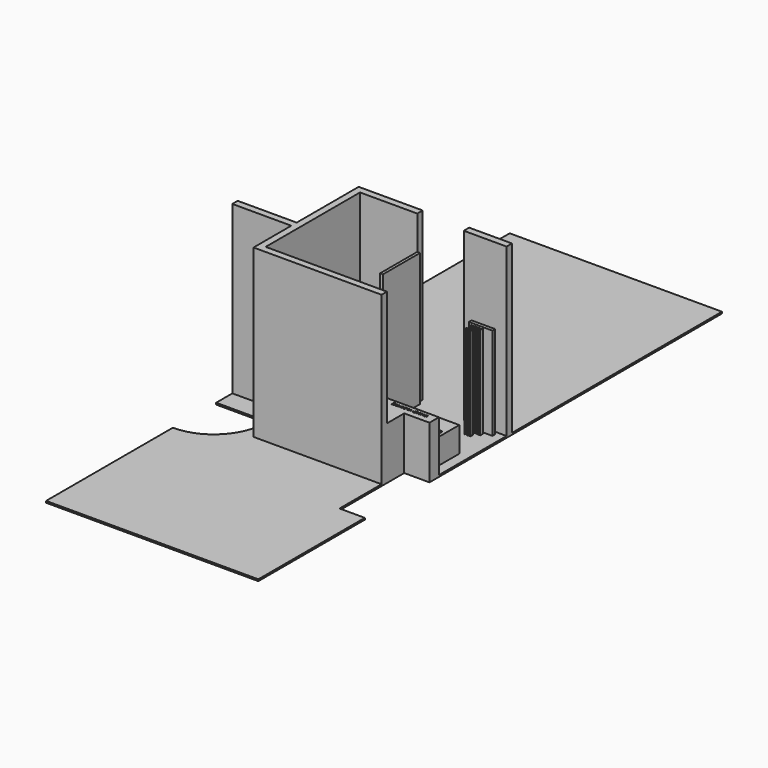
from build123d import *

# Parameters (mm, degrees)
F12_DEPTH    = 25
F5_W         = 800
F5_H         = 1700
F13_DEPTH    = 50
F6_W         = 365
F6_H         = 565
F14_DEPTH    = 400
F7_W         = 500
F7_H         = 500
F7_W_2       = 11.3769747938
F7_H_2       = 75.0792652576
F15_DEPTH    = 830
F8_W         = 5.7240140935
F8_H         = 37.7740814454
F16_DEPTH    = 780
F9_W         = 350
F9_H         = 50
F9_TEXT_SIZE = 67.0311508372
F17_DEPTH    = 1400
F18_DEPTH    = 20
F11_W        = 80
F11_H        = 80
F19_DEPTH    = 1000
F20_DEPTH    = 2500
F2_W         = 635
F2_H         = 100
F21_DEPTH    = 2500
F4_W         = 42
F4_H         = 690
F22_DEPTH    = 2000


# Not quite as in the source:
# - Text() gives the source's letters only with a copy of the font that has no kerning and outlines rounded to 1/6400 em; it was checked with that copy


with BuildPart() as f12:
    # F0 (on Top) → F12 (new body)
    with BuildSketch(Plane.XY):
        with BuildLine():
            Line((0, 3458.4132464471), (0, 1108.5698489868))
            Line((0, 1108.5698489868), (3150, 1108.5698489868))
            Line((3150, 1108.5698489868), (3150, 3083.5698489868))
            Line((3150, 3083.5698489868), (2775, 3083.5698489868))
            Line((2775, 3083.5698489868), (2775, 4283.5698489868))
            Line((2775, 4283.5698489868), (3150, 4283.5698489868))
            Line((3150, 4283.5698489868), (3150, 9708.5698489868))
            Line((3150, 9708.5698489868), (0, 9708.5698489868))
            Line((0, 9708.5698489868), (0, 7088.5698489868))
            Line((0, 7088.5698489868), (125, 7088.5698489868))
            Line((125, 7088.5698489868), (125, 6363.5698489868))
            Line((125, 6363.5698489868), (0, 6363.5698489868))
            Line((0, 6363.5698489868), (0, 5725.5698489868))
            ThreePointArc((0, 5725.5698489868), (523.7556682271, 5517.0352950627), (760.8416392391, 5005.5698489868))
            Line((760.8416392391, 5005.5698489868), (762, 5005.5698489868))
            Line((762, 5005.5698489868), (762, 4963.5698489868))
            Line((762, 4963.5698489868), (0, 4963.5698489868))
            Line((0, 4963.5698489868), (0, 4263.5698489868))
            Line((0, 4263.5698489868), (762, 4263.5698489868))
            ThreePointArc((762, 4263.5698489868), (554.2835814394, 3696.9960111463), (0, 3458.4132464471))
        make_face()
    extrude(amount=F12_DEPTH)

    # F5 (on Top) → F13 (join)
    with BuildSketch(Plane.XY):
        with Locations((1395, 4833.5698489868)):
            Rectangle(F5_W, F5_H)
        with BuildLine():
            add(Edge.make_bspline(
                [(1105.7062591253, 4987.2192112614), (1109.4488119877, 4983.0056568482), (1115.9664550678, 4983.0056568482)],
                knots=[0, 0, 0, 1, 1, 1], degree=2))
            add(Edge.make_bspline(
                [(1115.9664550678, 4983.0056568482), (1119.4798720407, 4983.0056568482), (1122.7386935808, 4983.5148477139)],
                knots=[0, 0, 0, 1, 1, 1], degree=2))
            add(Edge.make_bspline(
                [(1122.7386935808, 4983.5148477139), (1125.9975151209, 4984.0240385795), (1127.906980867, 4984.5841485317)],
                knots=[0, 0, 0, 1, 1, 1], degree=2))
            Line((1127.906980867, 4984.5841485317), (1127.906980867, 4974.4767098488))
            add(Edge.make_bspline(
                [(1127.906980867, 4974.4767098488), (1125.7683792313, 4973.4583281176), (1121.5930141331, 4972.7709204489)],
                knots=[0, 0, 0, 1, 1, 1], degree=2))
            add(Edge.make_bspline(
                [(1121.5930141331, 4972.7709204489), (1117.4176490349, 4972.0835127803), (1114.0569893217, 4972.0835127803)],
                knots=[0, 0, 0, 1, 1, 1], degree=2))
            add(Edge.make_bspline(
                [(1114.0569893217, 4972.0835127803), (1088.7756628428, 4972.0835127803), (1088.7756628428, 4998.7396545964)],
                knots=[0, 0, 0, 1, 1, 1], degree=2))
            Line((1088.7756628428, 4998.7396545964), (1088.7756628428, 5050.6262038048))
            Line((1088.7756628428, 5050.6262038048), (1076.2750270915, 5050.6262038048))
            Line((1076.2750270915, 5050.6262038048), (1076.2750270915, 5056.9910896252))
            Line((1076.2750270915, 5056.9910896252), (1088.7756628428, 5062.4903509741))
            Line((1088.7756628428, 5062.4903509741), (1094.3258432783, 5081.1012771131))
            Line((1094.3258432783, 5081.1012771131), (1101.9637062628, 5081.1012771131))
            Line((1101.9637062628, 5081.1012771131), (1101.9637062628, 5060.8863997474))
            Line((1101.9637062628, 5060.8863997474), (1127.270492285, 5060.8863997474))
            Line((1127.270492285, 5060.8863997474), (1127.270492285, 5050.6262038048))
            Line((1127.270492285, 5050.6262038048), (1101.9637062628, 5050.6262038048))
            Line((1101.9637062628, 5050.6262038048), (1101.9637062628, 4999.2997645486))
            add(Edge.make_bspline(
                [(1101.9637062628, 4999.2997645486), (1101.9637062628, 4991.4327656745), (1105.7062591253, 4987.2192112614)],
                knots=[0, 0, 0, 1, 1, 1], degree=2))
        make_face(mode=Mode.SUBTRACT)
        with BuildLine():
            add(Edge.make_bspline(
                [(1170.0679845417, 5057.8694438685), (1176.9166016845, 5062.4903509741), (1185.1145746213, 5062.4903509741)],
                knots=[0, 0, 0, 1, 1, 1], degree=2))
            add(Edge.make_bspline(
                [(1185.1145746213, 5062.4903509741), (1190.9193504895, 5062.4903509741), (1195.5275278236, 5061.5228883294)],
                knots=[0, 0, 0, 1, 1, 1], degree=2))
            Line((1195.5275278236, 5061.5228883294), (1193.6944407073, 5049.2768480108))
            add(Edge.make_bspline(
                [(1193.6944407073, 5049.2768480108), (1188.2970175315, 5050.4734465451), (1184.1471119766, 5050.4734465451)],
                knots=[0, 0, 0, 1, 1, 1], degree=2))
            add(Edge.make_bspline(
                [(1184.1471119766, 5050.4734465451), (1173.5559419713, 5050.4734465451), (1166.0453767032, 5041.8808506875)],
                knots=[0, 0, 0, 1, 1, 1], degree=2))
            add(Edge.make_bspline(
                [(1166.0453767032, 5041.8808506875), (1158.5348114351, 5033.2882548299), (1158.5348114351, 5020.4821045591)],
                knots=[0, 0, 0, 1, 1, 1], degree=2))
            Line((1158.5348114351, 5020.4821045591), (1158.5348114351, 4973.6874640071))
            Line((1158.5348114351, 4973.6874640071), (1145.3213084718, 4973.6874640071))
            Line((1145.3213084718, 4973.6874640071), (1145.3213084718, 5060.8863997474))
            Line((1145.3213084718, 5060.8863997474), (1156.2179929964, 5060.8863997474))
            Line((1156.2179929964, 5060.8863997474), (1157.7455655933, 5044.7450493067))
            Line((1157.7455655933, 5044.7450493067), (1158.3820541754, 5044.7450493067))
            add(Edge.make_bspline(
                [(1158.3820541754, 5044.7450493067), (1163.2193673989, 5053.2485367628), (1170.0679845417, 5057.8694438685)],
                knots=[0, 0, 0, 1, 1, 1], degree=2))
        make_face(mode=Mode.SUBTRACT)
        with BuildLine():
            add(Edge.make_bspline(
                [(1138.5999890454, 5233.4766436549), (1144.0483313077, 5227.7482464165), (1144.0483313077, 5219.0665421574)],
                knots=[0, 0, 0, 1, 1, 1], degree=2))
            add(Edge.make_bspline(
                [(1144.0483313077, 5219.0665421574), (1144.0483313077, 5206.8968804686), (1134.9847338994, 5200.290128987)],
                knots=[0, 0, 0, 1, 1, 1], degree=2))
            add(Edge.make_bspline(
                [(1134.9847338994, 5200.290128987), (1125.921136491, 5193.6833775054), (1109.5251906175, 5193.6833775054)],
                knots=[0, 0, 0, 1, 1, 1], degree=2))
            add(Edge.make_bspline(
                [(1109.5251906175, 5193.6833775054), (1092.1872416426, 5193.6833775054), (1082.4871556522, 5199.1826388543)],
                knots=[0, 0, 0, 1, 1, 1], degree=2))
            Line((1082.4871556522, 5199.1826388543), (1082.4871556522, 5211.4286791728))
            add(Edge.make_bspline(
                [(1082.4871556522, 5211.4286791728), (1088.7756628428, 5208.2462362626), (1095.96798382, 5206.4258789179)],
                knots=[0, 0, 0, 1, 1, 1], degree=2))
            add(Edge.make_bspline(
                [(1095.96798382, 5206.4258789179), (1103.1603047971, 5204.6055215733), (1109.8561646802, 5204.6055215733)],
                knots=[0, 0, 0, 1, 1, 1], degree=2))
            add(Edge.make_bspline(
                [(1109.8561646802, 5204.6055215733), (1120.1927392526, 5204.6055215733), (1125.7556494597, 5207.9025324283)],
                knots=[0, 0, 0, 1, 1, 1], degree=2))
            add(Edge.make_bspline(
                [(1125.7556494597, 5207.9025324283), (1131.3185596668, 5211.1995432833), (1131.3185596668, 5217.9717817962)],
                knots=[0, 0, 0, 1, 1, 1], degree=2))
            add(Edge.make_bspline(
                [(1131.3185596668, 5217.9717817962), (1131.3185596668, 5223.0636904526), (1126.914058679, 5226.6789455986)],
                knots=[0, 0, 0, 1, 1, 1], degree=2))
            add(Edge.make_bspline(
                [(1126.914058679, 5226.6789455986), (1122.5095576913, 5230.2942007446), (1109.6779478772, 5235.2333521413)],
                knots=[0, 0, 0, 1, 1, 1], degree=2))
            add(Edge.make_bspline(
                [(1109.6779478772, 5235.2333521413), (1097.5082861885, 5239.7651508455), (1092.3781882172, 5243.151270102)],
                knots=[0, 0, 0, 1, 1, 1], degree=2))
            add(Edge.make_bspline(
                [(1092.3781882172, 5243.151270102), (1087.2480902459, 5246.5373893585), (1084.7403252327, 5250.8273224014)],
                knots=[0, 0, 0, 1, 1, 1], degree=2))
            add(Edge.make_bspline(
                [(1084.7403252327, 5250.8273224014), (1082.2325602194, 5255.1172554444), (1082.2325602194, 5261.0747885724)],
                knots=[0, 0, 0, 1, 1, 1], degree=2))
            add(Edge.make_bspline(
                [(1082.2325602194, 5261.0747885724), (1082.2325602194, 5271.7423372075), (1090.9142644785, 5277.9162764533)],
                knots=[0, 0, 0, 1, 1, 1], degree=2))
            add(Edge.make_bspline(
                [(1090.9142644785, 5277.9162764533), (1099.5959687376, 5284.0902156992), (1114.6934779037, 5284.0902156992)],
                knots=[0, 0, 0, 1, 1, 1], degree=2))
            add(Edge.make_bspline(
                [(1114.6934779037, 5284.0902156992), (1128.7726053386, 5284.0902156992), (1142.2407037347, 5278.3618184607)],
                knots=[0, 0, 0, 1, 1, 1], degree=2))
            Line((1142.2407037347, 5278.3618184607), (1137.5306882275, 5267.6178911958))
            add(Edge.make_bspline(
                [(1137.5306882275, 5267.6178911958), (1124.4190234374, 5273.0153143716), (1113.7514748023, 5273.0153143716)],
                knots=[0, 0, 0, 1, 1, 1], degree=2))
            add(Edge.make_bspline(
                [(1113.7514748023, 5273.0153143716), (1104.3569033313, 5273.0153143716), (1099.583238966, 5270.0747371225)],
                knots=[0, 0, 0, 1, 1, 1], degree=2))
            add(Edge.make_bspline(
                [(1099.583238966, 5270.0747371225), (1094.8095746006, 5267.1341598735), (1094.8095746006, 5261.9658725872)],
                knots=[0, 0, 0, 1, 1, 1], degree=2))
            add(Edge.make_bspline(
                [(1094.8095746006, 5261.9658725872), (1094.8095746006, 5258.4524556144), (1096.604472402, 5255.9956096877)],
                knots=[0, 0, 0, 1, 1, 1], degree=2))
            add(Edge.make_bspline(
                [(1096.604472402, 5255.9956096877), (1098.3993702034, 5253.538763761), (1102.3710589553, 5251.3110537238)],
                knots=[0, 0, 0, 1, 1, 1], degree=2))
            add(Edge.make_bspline(
                [(1102.3710589553, 5251.3110537238), (1106.3427477073, 5249.0833436866), (1117.6467849244, 5244.8570595019)],
                knots=[0, 0, 0, 1, 1, 1], degree=2))
            add(Edge.make_bspline(
                [(1117.6467849244, 5244.8570595019), (1133.1516467831, 5239.2050408933), (1138.5999890454, 5233.4766436549)],
                knots=[0, 0, 0, 1, 1, 1], degree=2))
        make_face(mode=Mode.SUBTRACT)
        with BuildLine():
            Line((1275.2668173822, 4973.6874640071), (1265.4648932187, 4973.6874640071))
            Line((1265.4648932187, 4973.6874640071), (1262.8425602607, 4986.1117211286))
            Line((1262.8425602607, 4986.1117211286), (1262.2060716787, 4986.1117211286))
            add(Edge.make_bspline(
                [(1262.2060716787, 4986.1117211286), (1255.6884285985, 4977.9137481919), (1249.2089748333, 4974.9986304861)],
                knots=[0, 0, 0, 1, 1, 1], degree=2))
            add(Edge.make_bspline(
                [(1249.2089748333, 4974.9986304861), (1242.7295210681, 4972.0835127803), (1233.0039755344, 4972.0835127803)],
                knots=[0, 0, 0, 1, 1, 1], degree=2))
            add(Edge.make_bspline(
                [(1233.0039755344, 4972.0835127803), (1220.045068004, 4972.0835127803), (1212.6872599955, 4978.7793726635)],
                knots=[0, 0, 0, 1, 1, 1], degree=2))
            add(Edge.make_bspline(
                [(1212.6872599955, 4978.7793726635), (1205.3294519871, 4985.4752325466), (1205.3294519871, 4997.797651495)],
                knots=[0, 0, 0, 1, 1, 1], degree=2))
            add(Edge.make_bspline(
                [(1205.3294519871, 4997.797651495), (1205.3294519871, 5024.1991978782), (1247.5668342916, 5025.4721750423)],
                knots=[0, 0, 0, 1, 1, 1], degree=2))
            Line((1247.5668342916, 5025.4721750423), (1262.3588289384, 5025.9559063647))
            Line((1262.3588289384, 5025.9559063647), (1262.3588289384, 5031.3787890837))
            add(Edge.make_bspline(
                [(1262.3588289384, 5031.3787890837), (1262.3588289384, 5041.6389850263), (1257.9543279506, 5046.5272173364)],
                knots=[0, 0, 0, 1, 1, 1], degree=2))
            add(Edge.make_bspline(
                [(1257.9543279506, 5046.5272173364), (1253.5498269628, 5051.4154496465), (1243.8242814292, 5051.4154496465)],
                knots=[0, 0, 0, 1, 1, 1], degree=2))
            add(Edge.make_bspline(
                [(1243.8242814292, 5051.4154496465), (1232.9275969046, 5051.4154496465), (1219.1794435324, 5044.7450493067)],
                knots=[0, 0, 0, 1, 1, 1], degree=2))
            Line((1219.1794435324, 5044.7450493067), (1215.1059166073, 5054.8524879896))
            add(Edge.make_bspline(
                [(1215.1059166073, 5054.8524879896), (1221.5471810576, 5058.3404454192), (1229.2232333571, 5060.3262897952)],
                knots=[0, 0, 0, 1, 1, 1], degree=2))
            add(Edge.make_bspline(
                [(1229.2232333571, 5060.3262897952), (1236.8992856565, 5062.3121341711), (1244.6389868142, 5062.3121341711)],
                knots=[0, 0, 0, 1, 1, 1], degree=2))
            add(Edge.make_bspline(
                [(1244.6389868142, 5062.3121341711), (1260.2202273027, 5062.3121341711), (1267.7435223425, 5055.3998681701)],
                knots=[0, 0, 0, 1, 1, 1], degree=2))
            add(Edge.make_bspline(
                [(1267.7435223425, 5055.3998681701), (1275.2668173822, 5048.4876021691), (1275.2668173822, 5033.2118762)],
                knots=[0, 0, 0, 1, 1, 1], degree=2))
            Line((1275.2668173822, 5033.2118762), (1275.2668173822, 4973.6874640071))
        make_face(mode=Mode.SUBTRACT)
        with BuildLine():
            Line((1323.7927068774, 4973.2037326847), (1288.6076180619, 5060.8863997474))
            Line((1288.6076180619, 5060.8863997474), (1302.7885836699, 5060.8863997474))
            Line((1302.7885836699, 5060.8863997474), (1321.8832411313, 5011.1639117179))
            add(Edge.make_bspline(
                [(1321.8832411313, 5011.1639117179), (1328.1462887786, 4994.1314772624), (1329.6738613755, 4986.5699929077)],
                knots=[0, 0, 0, 1, 1, 1], degree=2))
            Line((1329.6738613755, 4986.5699929077), (1330.3103499576, 4986.5699929077))
            add(Edge.make_bspline(
                [(1330.3103499576, 4986.5699929077), (1331.3287316888, 4990.6435198328), (1334.6384723155, 5000.4709035396)],
                knots=[0, 0, 0, 1, 1, 1], degree=2))
            add(Edge.make_bspline(
                [(1334.6384723155, 5000.4709035396), (1337.9482129421, 5010.2982872464), (1356.2536245617, 5060.8863997474)],
                knots=[0, 0, 0, 1, 1, 1], degree=2))
            Line((1356.2536245617, 5060.8863997474), (1370.4091306264, 5060.8863997474))
            Line((1370.4091306264, 5060.8863997474), (1332.9326829156, 4961.5941809482))
            add(Edge.make_bspline(
                [(1332.9326829156, 4961.5941809482), (1327.3570429369, 4946.8785649313), (1319.9228562986, 4940.7046256855)],
                knots=[0, 0, 0, 1, 1, 1], degree=2))
            add(Edge.make_bspline(
                [(1319.9228562986, 4940.7046256855), (1312.4886696603, 4934.5306864396), (1301.6683637655, 4934.5306864396)],
                knots=[0, 0, 0, 1, 1, 1], degree=2))
            add(Edge.make_bspline(
                [(1301.6683637655, 4934.5306864396), (1295.6089924644, 4934.5306864396), (1289.7278379663, 4935.9055017769)],
                knots=[0, 0, 0, 1, 1, 1], degree=2))
            Line((1289.7278379663, 4935.9055017769), (1289.7278379663, 4946.4712122388))
            add(Edge.make_bspline(
                [(1289.7278379663, 4946.4712122388), (1294.1068794108, 4945.5292091374), (1299.5043025865, 4945.5292091374)],
                knots=[0, 0, 0, 1, 1, 1], degree=2))
            add(Edge.make_bspline(
                [(1299.5043025865, 4945.5292091374), (1313.1251582423, 4945.5292091374), (1318.9299341106, 4960.8049351065)],
                knots=[0, 0, 0, 1, 1, 1], degree=2))
            Line((1318.9299341106, 4960.8049351065), (1323.7927068774, 4973.2037326847))
        make_face(mode=Mode.SUBTRACT)
        with BuildLine():
            Line((1238.4268582534, 5195.2873287321), (1225.2133552902, 5195.2873287321))
            Line((1225.2133552902, 5195.2873287321), (1225.2133552902, 5251.7056766447))
            add(Edge.make_bspline(
                [(1225.2133552902, 5251.7056766447), (1225.2133552902, 5262.3477657365), (1220.363312295, 5267.6051614242)],
                knots=[0, 0, 0, 1, 1, 1], degree=2))
            add(Edge.make_bspline(
                [(1220.363312295, 5267.6051614242), (1215.5132692998, 5272.8625571119), (1205.1512351841, 5272.8625571119)],
                knots=[0, 0, 0, 1, 1, 1], degree=2))
            add(Edge.make_bspline(
                [(1205.1512351841, 5272.8625571119), (1191.4030818119, 5272.8625571119), (1185.0763853064, 5265.377451387)],
                knots=[0, 0, 0, 1, 1, 1], degree=2))
            add(Edge.make_bspline(
                [(1185.0763853064, 5265.377451387), (1178.7496888008, 5257.8923456622), (1178.7496888008, 5240.8853707499)],
                knots=[0, 0, 0, 1, 1, 1], degree=2))
            Line((1178.7496888008, 5240.8853707499), (1178.7496888008, 5195.2873287321))
            Line((1178.7496888008, 5195.2873287321), (1165.5361858376, 5195.2873287321))
            Line((1165.5361858376, 5195.2873287321), (1165.5361858376, 5319.0970877117))
            Line((1165.5361858376, 5319.0970877117), (1178.7496888008, 5319.0970877117))
            Line((1178.7496888008, 5319.0970877117), (1178.7496888008, 5281.6206400008))
            add(Edge.make_bspline(
                [(1178.7496888008, 5281.6206400008), (1178.7496888008, 5274.8484014879), (1178.1132002188, 5270.3929814135)],
                knots=[0, 0, 0, 1, 1, 1], degree=2))
            Line((1178.1132002188, 5270.3929814135), (1178.9024460605, 5270.3929814135))
            add(Edge.make_bspline(
                [(1178.9024460605, 5270.3929814135), (1182.7977561826, 5276.6814886041), (1190.0028069314, 5280.2967437502)],
                knots=[0, 0, 0, 1, 1, 1], degree=2))
            add(Edge.make_bspline(
                [(1190.0028069314, 5280.2967437502), (1197.2078576802, 5283.9119988962), (1206.4242123482, 5283.9119988962)],
                knots=[0, 0, 0, 1, 1, 1], degree=2))
            add(Edge.make_bspline(
                [(1206.4242123482, 5283.9119988962), (1222.4128055292, 5283.9119988962), (1230.4198318913, 5276.3123252266)],
                knots=[0, 0, 0, 1, 1, 1], degree=2))
            add(Edge.make_bspline(
                [(1230.4198318913, 5276.3123252266), (1238.4268582534, 5268.7126515569), (1238.4268582534, 5252.1639484237)],
                knots=[0, 0, 0, 1, 1, 1], degree=2))
            Line((1238.4268582534, 5252.1639484237), (1238.4268582534, 5195.2873287321))
        make_face(mode=Mode.SUBTRACT)
        with BuildLine():
            add(Edge.make_bspline(
                [(1330.0175652098, 5271.9078242388), (1340.7996817897, 5259.7254327784), (1340.7996817897, 5238.9759050038)],
                knots=[0, 0, 0, 1, 1, 1], degree=2))
            add(Edge.make_bspline(
                [(1340.7996817897, 5238.9759050038), (1340.7996817897, 5217.6408077336), (1330.0684842964, 5205.6620926195)],
                knots=[0, 0, 0, 1, 1, 1], degree=2))
            add(Edge.make_bspline(
                [(1330.0684842964, 5205.6620926195), (1319.3372868031, 5193.6833775054), (1300.3953866014, 5193.6833775054)],
                knots=[0, 0, 0, 1, 1, 1], degree=2))
            add(Edge.make_bspline(
                [(1300.3953866014, 5193.6833775054), (1288.6839966918, 5193.6833775054), (1279.6203992834, 5199.1826388543)],
                knots=[0, 0, 0, 1, 1, 1], degree=2))
            add(Edge.make_bspline(
                [(1279.6203992834, 5199.1826388543), (1270.5568018751, 5204.6819002031), (1265.6176504784, 5214.9420961457)],
                knots=[0, 0, 0, 1, 1, 1], degree=2))
            add(Edge.make_bspline(
                [(1265.6176504784, 5214.9420961457), (1260.6784990818, 5225.2022920883), (1260.6784990818, 5238.9759050038)],
                knots=[0, 0, 0, 1, 1, 1], degree=2))
            add(Edge.make_bspline(
                [(1260.6784990818, 5238.9759050038), (1260.6784990818, 5260.2855427306), (1271.3460477168, 5272.1878792149)],
                knots=[0, 0, 0, 1, 1, 1], degree=2))
            add(Edge.make_bspline(
                [(1271.3460477168, 5272.1878792149), (1282.0135963519, 5284.0902156992), (1300.9554965536, 5284.0902156992)],
                knots=[0, 0, 0, 1, 1, 1], degree=2))
            add(Edge.make_bspline(
                [(1300.9554965536, 5284.0902156992), (1319.23544863, 5284.0902156992), (1330.0175652098, 5271.9078242388)],
                knots=[0, 0, 0, 1, 1, 1], degree=2))
        make_face(mode=Mode.SUBTRACT)
        with BuildLine():
            Line((1450.861287397, 5195.2873287321), (1435.1782087354, 5195.2873287321))
            Line((1435.1782087354, 5195.2873287321), (1419.1896155544, 5246.4355511853))
            add(Edge.make_bspline(
                [(1419.1896155544, 5246.4355511853), (1417.6620429575, 5251.1455666925), (1413.5375969459, 5267.7706484555)],
                knots=[0, 0, 0, 1, 1, 1], degree=2))
            Line((1413.5375969459, 5267.7706484555), (1412.9011083638, 5267.7706484555))
            add(Edge.make_bspline(
                [(1412.9011083638, 5267.7706484555), (1409.7186654536, 5253.8442782803), (1407.3254683851, 5246.2827939256)],
                knots=[0, 0, 0, 1, 1, 1], degree=2))
            Line((1407.3254683851, 5246.2827939256), (1390.8531438818, 5195.2873287321))
            Line((1390.8531438818, 5195.2873287321), (1375.5774179127, 5195.2873287321))
            Line((1375.5774179127, 5195.2873287321), (1351.7982044874, 5282.4862644724))
            Line((1351.7982044874, 5282.4862644724), (1365.6481960327, 5282.4862644724))
            add(Edge.make_bspline(
                [(1365.6481960327, 5282.4862644724), (1374.075304859, 5249.6179940956), (1378.4925356184, 5232.4328023803)],
                knots=[0, 0, 0, 1, 1, 1], degree=2))
            add(Edge.make_bspline(
                [(1378.4925356184, 5232.4328023803), (1382.9097663778, 5215.2476106651), (1383.5462549599, 5209.2900775371)],
                knots=[0, 0, 0, 1, 1, 1], degree=2))
            Line((1383.5462549599, 5209.2900775371), (1384.1827435419, 5209.2900775371))
            add(Edge.make_bspline(
                [(1384.1827435419, 5209.2900775371), (1385.0483680135, 5213.8218762413), (1386.9960230746, 5221.0269269901)],
                knots=[0, 0, 0, 1, 1, 1], degree=2))
            add(Edge.make_bspline(
                [(1386.9960230746, 5221.0269269901), (1388.9436781356, 5228.2319777388), (1390.3948721027, 5232.4328023803)],
                knots=[0, 0, 0, 1, 1, 1], degree=2))
            Line((1390.3948721027, 5232.4328023803), (1406.3834652837, 5282.4862644724))
            Line((1406.3834652837, 5282.4862644724), (1420.6917286081, 5282.4862644724))
            Line((1420.6917286081, 5282.4862644724), (1436.2984286398, 5232.4328023803))
            add(Edge.make_bspline(
                [(1436.2984286398, 5232.4328023803), (1440.7538487141, 5218.761027638), (1442.3323403976, 5209.4428347968)],
                knots=[0, 0, 0, 1, 1, 1], degree=2))
            Line((1442.3323403976, 5209.4428347968), (1442.9688289797, 5209.4428347968))
            add(Edge.make_bspline(
                [(1442.9688289797, 5209.4428347968), (1443.2998030423, 5212.3197631877), (1444.6873481512, 5218.2900260873)],
                knots=[0, 0, 0, 1, 1, 1], degree=2))
            add(Edge.make_bspline(
                [(1444.6873481512, 5218.2900260873), (1446.07489326, 5224.2602889869), (1461.2742405993, 5282.4862644724)],
                knots=[0, 0, 0, 1, 1, 1], degree=2))
            Line((1461.2742405993, 5282.4862644724), (1474.9460153416, 5282.4862644724))
            Line((1474.9460153416, 5282.4862644724), (1450.861287397, 5195.2873287321))
        make_face(mode=Mode.SUBTRACT)
        with BuildLine():
            add(Edge.make_bspline(
                [(1542.6174813847, 5195.007273756), (1536.3798932807, 5193.6833775054), (1527.5454317619, 5193.6833775054)],
                knots=[0, 0, 0, 1, 1, 1], degree=2))
            add(Edge.make_bspline(
                [(1527.5454317619, 5193.6833775054), (1508.221638411, 5193.6833775054), (1497.0321691386, 5205.4711460449)],
                knots=[0, 0, 0, 1, 1, 1], degree=2))
            add(Edge.make_bspline(
                [(1497.0321691386, 5205.4711460449), (1485.8426998663, 5217.2589145844), (1485.8426998663, 5238.1611996187)],
                knots=[0, 0, 0, 1, 1, 1], degree=2))
            add(Edge.make_bspline(
                [(1485.8426998663, 5238.1611996187), (1485.8426998663, 5259.2671609994), (1496.2301935252, 5271.6786883493)],
                knots=[0, 0, 0, 1, 1, 1], degree=2))
            add(Edge.make_bspline(
                [(1496.2301935252, 5271.6786883493), (1506.6176871842, 5284.0902156992), (1524.1338529621, 5284.0902156992)],
                knots=[0, 0, 0, 1, 1, 1], degree=2))
            add(Edge.make_bspline(
                [(1524.1338529621, 5284.0902156992), (1540.5043392923, 5284.0902156992), (1550.051668023, 5273.3080991193)],
                knots=[0, 0, 0, 1, 1, 1], degree=2))
            add(Edge.make_bspline(
                [(1550.051668023, 5273.3080991193), (1559.5989967537, 5262.5259825394), (1559.5989967537, 5244.8570595019)],
                knots=[0, 0, 0, 1, 1, 1], degree=2))
            Line((1559.5989967537, 5244.8570595019), (1559.5989967537, 5236.5063293054))
            Line((1559.5989967537, 5236.5063293054), (1499.5399341519, 5236.5063293054))
            add(Edge.make_bspline(
                [(1499.5399341519, 5236.5063293054), (1499.9472868444, 5221.1542247065), (1507.3050948528, 5213.1981174309)],
                knots=[0, 0, 0, 1, 1, 1], degree=2))
            add(Edge.make_bspline(
                [(1507.3050948528, 5213.1981174309), (1514.6629028613, 5205.2420101553), (1528.0291630843, 5205.2420101553)],
                knots=[0, 0, 0, 1, 1, 1], degree=2))
            add(Edge.make_bspline(
                [(1528.0291630843, 5205.2420101553), (1542.1082905191, 5205.2420101553), (1555.8564438913, 5211.1231646534)],
                knots=[0, 0, 0, 1, 1, 1], degree=2))
            Line((1555.8564438913, 5211.1231646534), (1555.8564438913, 5199.3353961139))
            add(Edge.make_bspline(
                [(1555.8564438913, 5199.3353961139), (1548.8550694888, 5196.3311700067), (1542.6174813847, 5195.007273756)],
                knots=[0, 0, 0, 1, 1, 1], degree=2))
        make_face(mode=Mode.SUBTRACT)
        with BuildLine():
            add(Edge.make_bspline(
                [(1606.8773686281, 5279.4693085935), (1613.7259857709, 5284.0902156992), (1621.9239587076, 5284.0902156992)],
                knots=[0, 0, 0, 1, 1, 1], degree=2))
            add(Edge.make_bspline(
                [(1621.9239587076, 5284.0902156992), (1627.7287345759, 5284.0902156992), (1632.3369119099, 5283.1227530544)],
                knots=[0, 0, 0, 1, 1, 1], degree=2))
            Line((1632.3369119099, 5283.1227530544), (1630.5038247936, 5270.8767127359))
            add(Edge.make_bspline(
                [(1630.5038247936, 5270.8767127359), (1625.1064016179, 5272.0733112701), (1620.9564960629, 5272.0733112701)],
                knots=[0, 0, 0, 1, 1, 1], degree=2))
            add(Edge.make_bspline(
                [(1620.9564960629, 5272.0733112701), (1610.3653260577, 5272.0733112701), (1602.8547607895, 5263.4807154125)],
                knots=[0, 0, 0, 1, 1, 1], degree=2))
            add(Edge.make_bspline(
                [(1602.8547607895, 5263.4807154125), (1595.3441955214, 5254.8881195549), (1595.3441955214, 5242.0819692841)],
                knots=[0, 0, 0, 1, 1, 1], degree=2))
            Line((1595.3441955214, 5242.0819692841), (1595.3441955214, 5195.2873287321))
            Line((1595.3441955214, 5195.2873287321), (1582.1306925581, 5195.2873287321))
            Line((1582.1306925581, 5195.2873287321), (1582.1306925581, 5282.4862644724))
            Line((1582.1306925581, 5282.4862644724), (1593.0273770828, 5282.4862644724))
            Line((1593.0273770828, 5282.4862644724), (1594.5549496797, 5266.3449140317))
            Line((1594.5549496797, 5266.3449140317), (1595.1914382617, 5266.3449140317))
            add(Edge.make_bspline(
                [(1595.1914382617, 5266.3449140317), (1600.0287514853, 5274.8484014879), (1606.8773686281, 5279.4693085935)],
                knots=[0, 0, 0, 1, 1, 1], degree=2))
        make_face(mode=Mode.SUBTRACT)
    extrude(amount=F13_DEPTH)

    # F6 (on Top) → F14 (join)
    with BuildSketch(Plane.XY):
        with Locations((2817.5, 4741.0698489868)):
            Rectangle(F6_W, F6_H)
        with BuildLine():
            Line((2854.6655345708, 4694.878578186), (2845.2522004437, 4694.878578186))
            Line((2845.2522004437, 4694.878578186), (2842.733827937, 4706.8102848199))
            Line((2842.733827937, 4706.8102848199), (2842.1225724742, 4706.8102848199))
            add(Edge.make_bspline(
                [(2842.1225724742, 4706.8102848199), (2835.8633165351, 4698.937314459), (2829.6407359238, 4696.1377644394)],
                knots=[0, 0, 0, 1, 1, 1], degree=2))
            add(Edge.make_bspline(
                [(2829.6407359238, 4696.1377644394), (2823.4181553125, 4693.3382144198), (2814.078171841, 4693.3382144198)],
                knots=[0, 0, 0, 1, 1, 1], degree=2))
            add(Edge.make_bspline(
                [(2814.078171841, 4693.3382144198), (2801.6330106184, 4693.3382144198), (2794.5668974684, 4699.7686218884)],
                knots=[0, 0, 0, 1, 1, 1], degree=2))
            add(Edge.make_bspline(
                [(2794.5668974684, 4699.7686218884), (2787.5007843185, 4706.1990293571), (2787.5007843185, 4718.0329351169)],
                knots=[0, 0, 0, 1, 1, 1], degree=2))
            add(Edge.make_bspline(
                [(2787.5007843185, 4718.0329351169), (2787.5007843185, 4743.3878117137), (2828.0636968298, 4744.6103226393)],
                knots=[0, 0, 0, 1, 1, 1], degree=2))
            Line((2828.0636968298, 4744.6103226393), (2842.2692737853, 4745.0748767911))
            Line((2842.2692737853, 4745.0748767911), (2842.2692737853, 4750.2827733341))
            add(Edge.make_bspline(
                [(2842.2692737853, 4750.2827733341), (2842.2692737853, 4760.1362113944), (2838.0393859827, 4764.8306533487)],
                knots=[0, 0, 0, 1, 1, 1], degree=2))
            add(Edge.make_bspline(
                [(2838.0393859827, 4764.8306533487), (2833.8094981801, 4769.525095303), (2824.4695147086, 4769.525095303)],
                knots=[0, 0, 0, 1, 1, 1], degree=2))
            add(Edge.make_bspline(
                [(2824.4695147086, 4769.525095303), (2814.0048211854, 4769.525095303), (2800.801703189, 4763.1191380529)],
                knots=[0, 0, 0, 1, 1, 1], degree=2))
            Line((2800.801703189, 4763.1191380529), (2796.8896682271, 4772.8258748021))
            add(Edge.make_bspline(
                [(2796.8896682271, 4772.8258748021), (2803.0755735106, 4776.1755547383), (2810.4473143919, 4778.0826717822)],
                knots=[0, 0, 0, 1, 1, 1], degree=2))
            add(Edge.make_bspline(
                [(2810.4473143919, 4778.0826717822), (2817.8190552733, 4779.9897888261), (2825.2519217009, 4779.9897888261)],
                knots=[0, 0, 0, 1, 1, 1], degree=2))
            add(Edge.make_bspline(
                [(2825.2519217009, 4779.9897888261), (2840.2154554302, 4779.9897888261), (2847.4404950005, 4773.3515545001)],
                knots=[0, 0, 0, 1, 1, 1], degree=2))
            add(Edge.make_bspline(
                [(2847.4404950005, 4773.3515545001), (2854.6655345708, 4766.7133201742), (2854.6655345708, 4752.043189067)],
                knots=[0, 0, 0, 1, 1, 1], degree=2))
            Line((2854.6655345708, 4752.043189067), (2854.6655345708, 4694.878578186))
        make_face(mode=Mode.SUBTRACT)
        with BuildLine():
            Line((2950.7793435413, 4694.878578186), (2938.0896801336, 4694.878578186))
            Line((2938.0896801336, 4694.878578186), (2938.0896801336, 4749.0602624085))
            add(Edge.make_bspline(
                [(2938.0896801336, 4749.0602624085), (2938.0896801336, 4759.2804537465), (2933.4319135071, 4764.3294238692)],
                knots=[0, 0, 0, 1, 1, 1], degree=2))
            add(Edge.make_bspline(
                [(2933.4319135071, 4764.3294238692), (2928.7741468805, 4769.378393992), (2918.8229079462, 4769.378393992)],
                knots=[0, 0, 0, 1, 1, 1], degree=2))
            add(Edge.make_bspline(
                [(2918.8229079462, 4769.378393992), (2905.6931406053, 4769.378393992), (2899.5805859773, 4762.2756055142)],
                knots=[0, 0, 0, 1, 1, 1], degree=2))
            add(Edge.make_bspline(
                [(2899.5805859773, 4762.2756055142), (2893.4680313493, 4755.1728170365), (2893.4680313493, 4738.815620852)],
                knots=[0, 0, 0, 1, 1, 1], degree=2))
            Line((2893.4680313493, 4738.815620852), (2893.4680313493, 4694.878578186))
            Line((2893.4680313493, 4694.878578186), (2880.7783679416, 4694.878578186))
            Line((2880.7783679416, 4694.878578186), (2880.7783679416, 4778.6205765895))
            Line((2880.7783679416, 4778.6205765895), (2891.0963601536, 4778.6205765895))
            Line((2891.0963601536, 4778.6205765895), (2893.1501785086, 4767.1534241074))
            Line((2893.1501785086, 4767.1534241074), (2893.7614339714, 4767.1534241074))
            add(Edge.make_bspline(
                [(2893.7614339714, 4767.1534241074), (2897.6734689333, 4773.3393293909), (2904.7029067555, 4776.7501348733)],
                knots=[0, 0, 0, 1, 1, 1], degree=2))
            add(Edge.make_bspline(
                [(2904.7029067555, 4776.7501348733), (2911.7323445777, 4780.1609403557), (2920.3632717124, 4780.1609403557)],
                knots=[0, 0, 0, 1, 1, 1], degree=2))
            add(Edge.make_bspline(
                [(2920.3632717124, 4780.1609403557), (2935.4979569713, 4780.1609403557), (2943.1386502563, 4772.8625501299)],
                knots=[0, 0, 0, 1, 1, 1], degree=2))
            add(Edge.make_bspline(
                [(2943.1386502563, 4772.8625501299), (2950.7793435413, 4765.5641599041), (2950.7793435413, 4749.5003663417)],
                knots=[0, 0, 0, 1, 1, 1], degree=2))
            Line((2950.7793435413, 4749.5003663417), (2950.7793435413, 4694.878578186))
        make_face(mode=Mode.SUBTRACT)
        with BuildLine():
            add(Edge.make_bspline(
                [(2730.4339743116, 4806.5916265671), (2772.292748404, 4806.5916265671), (2772.292748404, 4774.0483857277)],
                knots=[0, 0, 0, 1, 1, 1], degree=2))
            add(Edge.make_bspline(
                [(2772.292748404, 4774.0483857277), (2772.292748404, 4757.0799340804), (2760.7155699386, 4747.9477774662)],
                knots=[0, 0, 0, 1, 1, 1], degree=2))
            add(Edge.make_bspline(
                [(2760.7155699386, 4747.9477774662), (2749.1383914732, 4738.815620852), (2727.5977489642, 4738.815620852)],
                knots=[0, 0, 0, 1, 1, 1], degree=2))
            Line((2727.5977489642, 4738.815620852), (2714.4435314048, 4738.815620852))
            Line((2714.4435314048, 4738.815620852), (2714.4435314048, 4694.878578186))
            Line((2714.4435314048, 4694.878578186), (2701.4604653749, 4694.878578186))
            Line((2701.4604653749, 4694.878578186), (2701.4604653749, 4806.5916265671))
            Line((2701.4604653749, 4806.5916265671), (2730.4339743116, 4806.5916265671))
        make_face(mode=Mode.SUBTRACT)
    extrude(amount=F14_DEPTH)

    # F7 (on Top) → F15 (join)
    with BuildSketch(Plane.XY):
        with Locations((2095, 4213.5698489868)):
            Rectangle(F7_W, F7_H)
        with BuildLine():
            Line((1980.4324611194, 4205.9421539307), (1980.4324611194, 4306.0989898319))
            Line((1980.4324611194, 4306.0989898319), (2008.732411907, 4306.0989898319))
            add(Edge.make_bspline(
                [(2008.732411907, 4306.0989898319), (2028.6585585111, 4306.0989898319), (2037.5694260519, 4300.136490518)],
                knots=[0, 0, 0, 1, 1, 1], degree=2))
            add(Edge.make_bspline(
                [(2037.5694260519, 4300.136490518), (2046.4802935926, 4294.1739912041), (2046.4802935926, 4281.3063915819)],
                knots=[0, 0, 0, 1, 1, 1], degree=2))
            add(Edge.make_bspline(
                [(2046.4802935926, 4281.3063915819), (2046.4802935926, 4272.3845635644), (2041.5151976566, 4266.5974318774)],
                knots=[0, 0, 0, 1, 1, 1], degree=2))
            add(Edge.make_bspline(
                [(2041.5151976566, 4266.5974318774), (2036.5501017206, 4260.8103001904), (2027.0144870091, 4259.1004658283)],
                knots=[0, 0, 0, 1, 1, 1], degree=2))
            Line((2027.0144870091, 4259.1004658283), (2027.0144870091, 4258.4209162742))
            add(Edge.make_bspline(
                [(2027.0144870091, 4258.4209162742), (2049.8341994567, 4254.5189865761), (2049.8341994567, 4234.4393932985)],
                knots=[0, 0, 0, 1, 1, 1], degree=2))
            add(Edge.make_bspline(
                [(2049.8341994567, 4234.4393932985), (2049.8341994567, 4221.0237698423), (2040.7589247657, 4213.4829618865)],
                knots=[0, 0, 0, 1, 1, 1], degree=2))
            add(Edge.make_bspline(
                [(2040.7589247657, 4213.4829618865), (2031.6836500747, 4205.9421539307), (2015.374460775, 4205.9421539307)],
                knots=[0, 0, 0, 1, 1, 1], degree=2))
            Line((2015.374460775, 4205.9421539307), (1980.4324611194, 4205.9421539307))
        make_face(mode=Mode.SUBTRACT)
        with BuildLine():
            Line((2124.2339151601, 4205.9421539307), (2115.7943481166, 4205.9421539307))
            Line((2115.7943481166, 4205.9421539307), (2113.5364899205, 4216.6395791703))
            Line((2113.5364899205, 4216.6395791703), (2112.9884660865, 4216.6395791703))
            add(Edge.make_bspline(
                [(2112.9884660865, 4216.6395791703), (2107.3767020264, 4209.5810321884), (2101.7978193963, 4207.0710830287)],
                knots=[0, 0, 0, 1, 1, 1], degree=2))
            add(Edge.make_bspline(
                [(2101.7978193963, 4207.0710830287), (2096.2189367662, 4204.561133869), (2087.8451325827, 4204.561133869)],
                knots=[0, 0, 0, 1, 1, 1], degree=2))
            add(Edge.make_bspline(
                [(2087.8451325827, 4204.561133869), (2076.6873673225, 4204.561133869), (2070.3522118015, 4210.3263446026)],
                knots=[0, 0, 0, 1, 1, 1], degree=2))
            add(Edge.make_bspline(
                [(2070.3522118015, 4210.3263446026), (2064.0170562805, 4216.0915553363), (2064.0170562805, 4226.7012967625)],
                knots=[0, 0, 0, 1, 1, 1], degree=2))
            add(Edge.make_bspline(
                [(2064.0170562805, 4226.7012967625), (2064.0170562805, 4249.4333253966), (2100.3839179046, 4250.5293730646)],
                knots=[0, 0, 0, 1, 1, 1], degree=2))
            Line((2100.3839179046, 4250.5293730646), (2113.1199918066, 4250.9458711785))
            Line((2113.1199918066, 4250.9458711785), (2113.1199918066, 4255.6150342441))
            add(Edge.make_bspline(
                [(2113.1199918066, 4255.6150342441), (2113.1199918066, 4264.4491784482), (2109.3276668754, 4268.6580014932)],
                knots=[0, 0, 0, 1, 1, 1], degree=2))
            add(Edge.make_bspline(
                [(2109.3276668754, 4268.6580014932), (2105.5353419441, 4272.8668245383), (2097.1615377607, 4272.8668245383)],
                knots=[0, 0, 0, 1, 1, 1], degree=2))
            add(Edge.make_bspline(
                [(2097.1615377607, 4272.8668245383), (2087.7793697226, 4272.8668245383), (2075.9420549083, 4267.1235347581)],
                knots=[0, 0, 0, 1, 1, 1], degree=2))
            Line((2075.9420549083, 4267.1235347581), (2072.4347023707, 4275.8261532419))
            add(Edge.make_bspline(
                [(2072.4347023707, 4275.8261532419), (2077.9807035708, 4278.8293238522), (2084.5898710088, 4280.5391582143)],
                knots=[0, 0, 0, 1, 1, 1], degree=2))
            add(Edge.make_bspline(
                [(2084.5898710088, 4280.5391582143), (2091.1990384468, 4282.2489925764), (2097.8630082682, 4282.2489925764)],
                knots=[0, 0, 0, 1, 1, 1], degree=2))
            add(Edge.make_bspline(
                [(2097.8630082682, 4282.2489925764), (2111.2786317244, 4282.2489925764), (2117.7562734423, 4276.2974537392)],
                knots=[0, 0, 0, 1, 1, 1], degree=2))
            add(Edge.make_bspline(
                [(2117.7562734423, 4276.2974537392), (2124.2339151601, 4270.345914902), (2124.2339151601, 4257.193342886)],
                knots=[0, 0, 0, 1, 1, 1], degree=2))
            Line((2124.2339151601, 4257.193342886), (2124.2339151601, 4205.9421539307))
        make_face(mode=Mode.SUBTRACT)
        with BuildLine():
            add(Edge.make_bspline(
                [(2191.3777953014, 4238.8235839705), (2196.0688793204, 4233.8913694645), (2196.0688793204, 4226.4163243688)],
                knots=[0, 0, 0, 1, 1, 1], degree=2))
            add(Edge.make_bspline(
                [(2196.0688793204, 4226.4163243688), (2196.0688793204, 4215.9381086628), (2188.2650199243, 4210.2496212659)],
                knots=[0, 0, 0, 1, 1, 1], degree=2))
            add(Edge.make_bspline(
                [(2188.2650199243, 4210.2496212659), (2180.4611605282, 4204.561133869), (2166.3440665644, 4204.561133869)],
                knots=[0, 0, 0, 1, 1, 1], degree=2))
            add(Edge.make_bspline(
                [(2166.3440665644, 4204.561133869), (2151.4158973263, 4204.561133869), (2143.0640140962, 4209.2960597947)],
                knots=[0, 0, 0, 1, 1, 1], degree=2))
            Line((2143.0640140962, 4209.2960597947), (2143.0640140962, 4219.8400383608))
            add(Edge.make_bspline(
                [(2143.0640140962, 4219.8400383608), (2148.4784895761, 4217.0999191908), (2154.6711589003, 4215.5325710256)],
                knots=[0, 0, 0, 1, 1, 1], degree=2))
            add(Edge.make_bspline(
                [(2154.6711589003, 4215.5325710256), (2160.8638282244, 4213.9652228604), (2166.6290389581, 4213.9652228604)],
                knots=[0, 0, 0, 1, 1, 1], degree=2))
            add(Edge.make_bspline(
                [(2166.6290389581, 4213.9652228604), (2175.5289460222, 4213.9652228604), (2180.3186743313, 4216.8039863205)],
                knots=[0, 0, 0, 1, 1, 1], degree=2))
            add(Edge.make_bspline(
                [(2180.3186743313, 4216.8039863205), (2185.1084026405, 4219.6427497806), (2185.1084026405, 4225.4737233743)],
                knots=[0, 0, 0, 1, 1, 1], degree=2))
            add(Edge.make_bspline(
                [(2185.1084026405, 4225.4737233743), (2185.1084026405, 4229.8579140463), (2181.3160777092, 4232.9706894234)],
                knots=[0, 0, 0, 1, 1, 1], degree=2))
            add(Edge.make_bspline(
                [(2181.3160777092, 4232.9706894234), (2177.5237527779, 4236.0834648005), (2166.4755922846, 4240.3361297523)],
                knots=[0, 0, 0, 1, 1, 1], degree=2))
            add(Edge.make_bspline(
                [(2166.4755922846, 4240.3361297523), (2155.9973765785, 4244.2380594504), (2151.5803044765, 4247.1535462472)],
                knots=[0, 0, 0, 1, 1, 1], degree=2))
            add(Edge.make_bspline(
                [(2151.5803044765, 4247.1535462472), (2147.1632323745, 4250.0690330441), (2145.0040184686, 4253.7627136852)],
                knots=[0, 0, 0, 1, 1, 1], degree=2))
            add(Edge.make_bspline(
                [(2145.0040184686, 4253.7627136852), (2142.8448045626, 4257.4563943264), (2142.8448045626, 4262.5858974126)],
                knots=[0, 0, 0, 1, 1, 1], degree=2))
            add(Edge.make_bspline(
                [(2142.8448045626, 4262.5858974126), (2142.8448045626, 4271.7707768704), (2150.3198496583, 4277.0866080601)],
                knots=[0, 0, 0, 1, 1, 1], degree=2))
            add(Edge.make_bspline(
                [(2150.3198496583, 4277.0866080601), (2157.7948947541, 4282.4024392499), (2170.7940200965, 4282.4024392499)],
                knots=[0, 0, 0, 1, 1, 1], degree=2))
            add(Edge.make_bspline(
                [(2170.7940200965, 4282.4024392499), (2182.9163073045, 4282.4024392499), (2194.5124916318, 4277.4702247439)],
                knots=[0, 0, 0, 1, 1, 1], degree=2))
            Line((2194.5124916318, 4277.4702247439), (2190.4571152603, 4268.2195824261))
            add(Edge.make_bspline(
                [(2190.4571152603, 4268.2195824261), (2179.1678242799, 4272.8668245383), (2169.9829448221, 4272.8668245383)],
                knots=[0, 0, 0, 1, 1, 1], degree=2))
            add(Edge.make_bspline(
                [(2169.9829448221, 4272.8668245383), (2161.8941130324, 4272.8668245383), (2157.7839342774, 4270.3349544253)],
                knots=[0, 0, 0, 1, 1, 1], degree=2))
            add(Edge.make_bspline(
                [(2157.7839342774, 4270.3349544253), (2153.6737555224, 4267.8030843122), (2153.6737555224, 4263.3531307802)],
                knots=[0, 0, 0, 1, 1, 1], degree=2))
            add(Edge.make_bspline(
                [(2153.6737555224, 4263.3531307802), (2153.6737555224, 4260.3280392165), (2155.2191827343, 4258.2126672173)],
                knots=[0, 0, 0, 1, 1, 1], degree=2))
            add(Edge.make_bspline(
                [(2155.2191827343, 4258.2126672173), (2156.7646099461, 4256.097295218), (2160.1842786703, 4254.1792117991)],
                knots=[0, 0, 0, 1, 1, 1], degree=2))
            add(Edge.make_bspline(
                [(2160.1842786703, 4254.1792117991), (2163.6039473944, 4252.2611283801), (2173.3368506862, 4248.6222501223)],
                knots=[0, 0, 0, 1, 1, 1], degree=2))
            add(Edge.make_bspline(
                [(2173.3368506862, 4248.6222501223), (2186.6867112824, 4243.7557984764), (2191.3777953014, 4238.8235839705)],
                knots=[0, 0, 0, 1, 1, 1], degree=2))
        make_face(mode=Mode.SUBTRACT)
        with Locations((2220.258651353, 4243.4817865594)):
            Rectangle(F7_W_2, F7_H_2, mode=Mode.SUBTRACT)
        with BuildLine():
            Line((2312.8198769151, 4205.9421539307), (2301.4429021213, 4205.9421539307))
            Line((2301.4429021213, 4205.9421539307), (2301.4429021213, 4254.5189865761))
            add(Edge.make_bspline(
                [(2301.4429021213, 4254.5189865761), (2301.4429021213, 4263.6819450806), (2297.2669605062, 4268.2086219494)],
                knots=[0, 0, 0, 1, 1, 1], degree=2))
            add(Edge.make_bspline(
                [(2297.2669605062, 4268.2086219494), (2293.0910188912, 4272.7352988182), (2284.1691908737, 4272.7352988182)],
                knots=[0, 0, 0, 1, 1, 1], degree=2))
            add(Edge.make_bspline(
                [(2284.1691908737, 4272.7352988182), (2272.3976389195, 4272.7352988182), (2266.9174005795, 4266.3672618671)],
                knots=[0, 0, 0, 1, 1, 1], degree=2))
            add(Edge.make_bspline(
                [(2266.9174005795, 4266.3672618671), (2261.4371622395, 4259.9992249161), (2261.4371622395, 4245.3341071183)],
                knots=[0, 0, 0, 1, 1, 1], degree=2))
            Line((2261.4371622395, 4245.3341071183), (2261.4371622395, 4205.9421539307))
            Line((2261.4371622395, 4205.9421539307), (2250.0601874457, 4205.9421539307))
            Line((2250.0601874457, 4205.9421539307), (2250.0601874457, 4281.0214191882))
            Line((2250.0601874457, 4281.0214191882), (2259.3108297636, 4281.0214191882))
            Line((2259.3108297636, 4281.0214191882), (2261.1521898458, 4270.7404920624))
            Line((2261.1521898458, 4270.7404920624), (2261.7002136798, 4270.7404920624))
            add(Edge.make_bspline(
                [(2261.7002136798, 4270.7404920624), (2265.2075662174, 4276.2864932625), (2271.5098403084, 4279.3444662562)],
                knots=[0, 0, 0, 1, 1, 1], degree=2))
            add(Edge.make_bspline(
                [(2271.5098403084, 4279.3444662562), (2277.8121143993, 4282.4024392499), (2285.5502109354, 4282.4024392499)],
                knots=[0, 0, 0, 1, 1, 1], degree=2))
            add(Edge.make_bspline(
                [(2285.5502109354, 4282.4024392499), (2299.1192810651, 4282.4024392499), (2305.9695789901, 4275.859034672)],
                knots=[0, 0, 0, 1, 1, 1], degree=2))
            add(Edge.make_bspline(
                [(2305.9695789901, 4275.859034672), (2312.8198769151, 4269.315630094), (2312.8198769151, 4254.9135637366)],
                knots=[0, 0, 0, 1, 1, 1], degree=2))
            Line((2312.8198769151, 4254.9135637366), (2312.8198769151, 4205.9421539307))
        make_face(mode=Mode.SUBTRACT)
        with BuildLine():
            add(Edge.make_bspline(
                [(2215.5237254273, 4295.6426950792), (2213.6056420083, 4297.5278970682), (2213.6056420083, 4301.3640639062)],
                knots=[0, 0, 0, 1, 1, 1], degree=2))
            add(Edge.make_bspline(
                [(2213.6056420083, 4301.3640639062), (2213.6056420083, 4305.2659936042), (2215.5237254273, 4307.0854327331)],
                knots=[0, 0, 0, 1, 1, 1], degree=2))
            add(Edge.make_bspline(
                [(2215.5237254273, 4307.0854327331), (2217.4418088463, 4308.904871862), (2220.3353746898, 4308.904871862)],
                knots=[0, 0, 0, 1, 1, 1], degree=2))
            add(Edge.make_bspline(
                [(2220.3353746898, 4308.904871862), (2223.0754938597, 4308.904871862), (2225.0593401388, 4307.0525513031)],
                knots=[0, 0, 0, 1, 1, 1], degree=2))
            add(Edge.make_bspline(
                [(2225.0593401388, 4307.0525513031), (2227.0431864179, 4305.2002307441), (2227.0431864179, 4301.3640639062)],
                knots=[0, 0, 0, 1, 1, 1], degree=2))
            add(Edge.make_bspline(
                [(2227.0431864179, 4301.3640639062), (2227.0431864179, 4297.5278970682), (2225.0593401388, 4295.6426950792)],
                knots=[0, 0, 0, 1, 1, 1], degree=2))
            add(Edge.make_bspline(
                [(2225.0593401388, 4295.6426950792), (2223.0754938597, 4293.7574930903), (2220.3353746898, 4293.7574930903)],
                knots=[0, 0, 0, 1, 1, 1], degree=2))
            add(Edge.make_bspline(
                [(2220.3353746898, 4293.7574930903), (2217.4418088463, 4293.7574930903), (2215.5237254273, 4295.6426950792)],
                knots=[0, 0, 0, 1, 1, 1], degree=2))
        make_face(mode=Mode.SUBTRACT)
    extrude(amount=F15_DEPTH)

    # F8 (on Top) → F16 (join)
    with BuildSketch(Plane.XY):
        Polygon((3150, 4283.5698489868), (3150, 4458.5698489868), (2395, 4458.5698489868), (2395, 3963.5698489868), (2775, 3963.5698489868), (2775, 4283.5698489868), align=None)
        with BuildLine():
            Line((2516.7633179161, 4370.210647583), (2516.7633179161, 4420.6018236776))
            Line((2516.7633179161, 4420.6018236776), (2531.001665112, 4420.6018236776))
            add(Edge.make_bspline(
                [(2531.001665112, 4420.6018236776), (2541.0269614723, 4420.6018236776), (2545.5102210657, 4417.6019550198)],
                knots=[0, 0, 0, 1, 1, 1], degree=2))
            add(Edge.make_bspline(
                [(2545.5102210657, 4417.6019550198), (2549.9934806592, 4414.6020863619), (2549.9934806592, 4408.128105104)],
                knots=[0, 0, 0, 1, 1, 1], degree=2))
            add(Edge.make_bspline(
                [(2549.9934806592, 4408.128105104), (2549.9934806592, 4403.6393310461), (2547.4954282658, 4400.7276938193)],
                knots=[0, 0, 0, 1, 1, 1], degree=2))
            add(Edge.make_bspline(
                [(2547.4954282658, 4400.7276938193), (2544.9973758724, 4397.8160565926), (2540.1997918056, 4396.9558001392)],
                knots=[0, 0, 0, 1, 1, 1], degree=2))
            Line((2540.1997918056, 4396.9558001392), (2540.1997918056, 4396.6139033437))
            add(Edge.make_bspline(
                [(2540.1997918056, 4396.6139033437), (2551.6809067792, 4394.6507540014), (2551.6809067792, 4384.5482551389)],
                knots=[0, 0, 0, 1, 1, 1], degree=2))
            add(Edge.make_bspline(
                [(2551.6809067792, 4384.5482551389), (2551.6809067792, 4377.7985506588), (2547.1149302191, 4374.0045991209)],
                knots=[0, 0, 0, 1, 1, 1], degree=2))
            add(Edge.make_bspline(
                [(2547.1149302191, 4374.0045991209), (2542.548953659, 4370.210647583), (2534.3434305655, 4370.210647583)],
                knots=[0, 0, 0, 1, 1, 1], degree=2))
            Line((2534.3434305655, 4370.210647583), (2516.7633179161, 4370.210647583))
        make_face(mode=Mode.SUBTRACT)
        with BuildLine():
            add(Edge.make_bspline(
                [(2589.570791978, 4403.402209075), (2594.2415433625, 4398.1248666015), (2594.2415433625, 4389.1362895568)],
                knots=[0, 0, 0, 1, 1, 1], degree=2))
            add(Edge.make_bspline(
                [(2594.2415433625, 4389.1362895568), (2594.2415433625, 4379.8940471477), (2589.5928498358, 4374.7049361053)],
                knots=[0, 0, 0, 1, 1, 1], degree=2))
            add(Edge.make_bspline(
                [(2589.5928498358, 4374.7049361053), (2584.944156309, 4369.515825063), (2576.7386332154, 4369.515825063)],
                knots=[0, 0, 0, 1, 1, 1], degree=2))
            add(Edge.make_bspline(
                [(2576.7386332154, 4369.515825063), (2571.6653259264, 4369.515825063), (2567.7390272419, 4371.8980737031)],
                knots=[0, 0, 0, 1, 1, 1], degree=2))
            add(Edge.make_bspline(
                [(2567.7390272419, 4371.8980737031), (2563.8127285573, 4374.2803223431), (2561.6731163528, 4378.7249806854)],
                knots=[0, 0, 0, 1, 1, 1], degree=2))
            add(Edge.make_bspline(
                [(2561.6731163528, 4378.7249806854), (2559.5335041483, 4383.1696390278), (2559.5335041483, 4389.1362895568)],
                knots=[0, 0, 0, 1, 1, 1], degree=2))
            add(Edge.make_bspline(
                [(2559.5335041483, 4389.1362895568), (2559.5335041483, 4398.3675030371), (2564.1546253529, 4403.5235272927)],
                knots=[0, 0, 0, 1, 1, 1], degree=2))
            add(Edge.make_bspline(
                [(2564.1546253529, 4403.5235272927), (2568.7757465574, 4408.6795515484), (2576.981269651, 4408.6795515484)],
                knots=[0, 0, 0, 1, 1, 1], degree=2))
            add(Edge.make_bspline(
                [(2576.981269651, 4408.6795515484), (2584.9000405934, 4408.6795515484), (2589.570791978, 4403.402209075)],
                knots=[0, 0, 0, 1, 1, 1], degree=2))
        make_face(mode=Mode.SUBTRACT)
        Polygon((2599.5574870871, 4370.210647583), (2613.3767349852, 4389.5443599257), (2600.2412806782, 4407.9847290284), (2606.7593776517, 4407.9847290284), (2616.7185004387, 4393.5147743258), (2626.6445364389, 4407.9847290284), (2633.0964598391, 4407.9847290284), (2619.9610055321, 4389.5443599257), (2633.7802534302, 4370.210647583), (2627.3062721723, 4370.210647583), (2616.7185004387, 4385.5188008812), (2606.0314683451, 4370.210647583), align=None, mode=Mode.SUBTRACT)
        with BuildLine():
            add(Edge.make_bspline(
                [(2663.7458532221, 4370.0893293652), (2661.0437656442, 4369.515825063), (2657.2167273197, 4369.515825063)],
                knots=[0, 0, 0, 1, 1, 1], degree=2))
            add(Edge.make_bspline(
                [(2657.2167273197, 4369.515825063), (2648.8457702928, 4369.515825063), (2643.998556046, 4374.6222191387)],
                knots=[0, 0, 0, 1, 1, 1], degree=2))
            add(Edge.make_bspline(
                [(2643.998556046, 4374.6222191387), (2639.1513417992, 4379.7286132144), (2639.1513417992, 4388.7833638324)],
                knots=[0, 0, 0, 1, 1, 1], degree=2))
            add(Edge.make_bspline(
                [(2639.1513417992, 4388.7833638324), (2639.1513417992, 4397.9263458815), (2643.651144786, 4403.302948715)],
                knots=[0, 0, 0, 1, 1, 1], degree=2))
            add(Edge.make_bspline(
                [(2643.651144786, 4403.302948715), (2648.1509477728, 4408.6795515484), (2655.7388508485, 4408.6795515484)],
                knots=[0, 0, 0, 1, 1, 1], degree=2))
            add(Edge.make_bspline(
                [(2655.7388508485, 4408.6795515484), (2662.8304521243, 4408.6795515484), (2666.9663004577, 4404.0088001639)],
                knots=[0, 0, 0, 1, 1, 1], degree=2))
            add(Edge.make_bspline(
                [(2666.9663004577, 4404.0088001639), (2671.1021487912, 4399.3380487793), (2671.1021487912, 4391.6839721302)],
                knots=[0, 0, 0, 1, 1, 1], degree=2))
            Line((2671.1021487912, 4391.6839721302), (2671.1021487912, 4388.0664834546))
            Line((2671.1021487912, 4388.0664834546), (2645.0849055416, 4388.0664834546))
            add(Edge.make_bspline(
                [(2645.0849055416, 4388.0664834546), (2645.2613684038, 4381.4160393344), (2648.4487288528, 4377.9694990565)],
                knots=[0, 0, 0, 1, 1, 1], degree=2))
            add(Edge.make_bspline(
                [(2648.4487288528, 4377.9694990565), (2651.6360893018, 4374.5229587787), (2657.4262769686, 4374.5229587787)],
                knots=[0, 0, 0, 1, 1, 1], degree=2))
            add(Edge.make_bspline(
                [(2657.4262769686, 4374.5229587787), (2663.5252746443, 4374.5229587787), (2669.4808962444, 4377.0706413521)],
                knots=[0, 0, 0, 1, 1, 1], degree=2))
            Line((2669.4808962444, 4377.0706413521), (2669.4808962444, 4371.9642472764))
            add(Edge.make_bspline(
                [(2669.4808962444, 4371.9642472764), (2666.4479407999, 4370.6628336675), (2663.7458532221, 4370.0893293652)],
                knots=[0, 0, 0, 1, 1, 1], degree=2))
        make_face(mode=Mode.SUBTRACT)
        with BuildLine():
            Line((2707.3321801921, 4370.210647583), (2706.5711840987, 4375.2729259431))
            Line((2706.5711840987, 4375.2729259431), (2706.2623740898, 4375.2729259431))
            add(Edge.make_bspline(
                [(2706.2623740898, 4375.2729259431), (2702.3029886186, 4369.515825063), (2694.406275534, 4369.515825063)],
                knots=[0, 0, 0, 1, 1, 1], degree=2))
            add(Edge.make_bspline(
                [(2694.406275534, 4369.515825063), (2686.9948353204, 4369.515825063), (2682.8755303803, 4374.5836178876)],
                knots=[0, 0, 0, 1, 1, 1], degree=2))
            add(Edge.make_bspline(
                [(2682.8755303803, 4374.5836178876), (2678.7562254402, 4379.6514107121), (2678.7562254402, 4388.9929134813)],
                knots=[0, 0, 0, 1, 1, 1], degree=2))
            add(Edge.make_bspline(
                [(2678.7562254402, 4388.9929134813), (2678.7562254402, 4398.3344162504), (2682.8920737737, 4403.5069838994)],
                knots=[0, 0, 0, 1, 1, 1], degree=2))
            add(Edge.make_bspline(
                [(2682.8920737737, 4403.5069838994), (2687.0279221071, 4408.6795515484), (2694.406275534, 4408.6795515484)],
                knots=[0, 0, 0, 1, 1, 1], degree=2))
            add(Edge.make_bspline(
                [(2694.406275534, 4408.6795515484), (2702.0934389697, 4408.6795515484), (2706.1962005165, 4403.0878846016)],
                knots=[0, 0, 0, 1, 1, 1], degree=2))
            Line((2706.1962005165, 4403.0878846016), (2706.6483866009, 4403.0878846016))
            Line((2706.6483866009, 4403.0878846016), (2706.4057501654, 4405.8120300372))
            Line((2706.4057501654, 4405.8120300372), (2706.2623740898, 4408.4700018995))
            Line((2706.2623740898, 4408.4700018995), (2706.2623740898, 4423.844328771))
            Line((2706.2623740898, 4423.844328771), (2711.9863881833, 4423.844328771))
            Line((2711.9863881833, 4423.844328771), (2711.9863881833, 4370.210647583))
            Line((2711.9863881833, 4370.210647583), (2707.3321801921, 4370.210647583))
        make_face(mode=Mode.SUBTRACT)
        with Locations((2745.3213257508, 4389.0976883057)):
            Rectangle(F8_W, F8_H, mode=Mode.SUBTRACT)
        with BuildLine():
            add(Edge.make_bspline(
                [(2742.9390771108, 4415.3410245975), (2741.974045833, 4416.289512482), (2741.974045833, 4418.2195750376)],
                knots=[0, 0, 0, 1, 1, 1], degree=2))
            add(Edge.make_bspline(
                [(2741.974045833, 4418.2195750376), (2741.974045833, 4420.1827243798), (2742.9390771108, 4421.0981254776)],
                knots=[0, 0, 0, 1, 1, 1], degree=2))
            add(Edge.make_bspline(
                [(2742.9390771108, 4421.0981254776), (2743.9041083886, 4422.0135265754), (2745.3599270019, 4422.0135265754)],
                knots=[0, 0, 0, 1, 1, 1], degree=2))
            add(Edge.make_bspline(
                [(2745.3599270019, 4422.0135265754), (2746.7385431131, 4422.0135265754), (2747.7366611775, 4421.0815820843)],
                knots=[0, 0, 0, 1, 1, 1], degree=2))
            add(Edge.make_bspline(
                [(2747.7366611775, 4421.0815820843), (2748.734779242, 4420.1496375932), (2748.734779242, 4418.2195750376)],
                knots=[0, 0, 0, 1, 1, 1], degree=2))
            add(Edge.make_bspline(
                [(2748.734779242, 4418.2195750376), (2748.734779242, 4416.289512482), (2747.7366611775, 4415.3410245975)],
                knots=[0, 0, 0, 1, 1, 1], degree=2))
            add(Edge.make_bspline(
                [(2747.7366611775, 4415.3410245975), (2746.7385431131, 4414.392536713), (2745.3599270019, 4414.392536713)],
                knots=[0, 0, 0, 1, 1, 1], degree=2))
            add(Edge.make_bspline(
                [(2745.3599270019, 4414.392536713), (2743.9041083886, 4414.392536713), (2742.9390771108, 4415.3410245975)],
                knots=[0, 0, 0, 1, 1, 1], degree=2))
        make_face(mode=Mode.SUBTRACT)
        with BuildLine():
            Line((2791.8909779853, 4370.210647583), (2786.1669638919, 4370.210647583))
            Line((2786.1669638919, 4370.210647583), (2786.1669638919, 4394.6507540014))
            add(Edge.make_bspline(
                [(2786.1669638919, 4394.6507540014), (2786.1669638919, 4399.2608462771), (2784.0659529385, 4401.5383200927)],
                knots=[0, 0, 0, 1, 1, 1], degree=2))
            add(Edge.make_bspline(
                [(2784.0659529385, 4401.5383200927), (2781.9649419851, 4403.8157939083), (2777.4761679272, 4403.8157939083)],
                knots=[0, 0, 0, 1, 1, 1], degree=2))
            add(Edge.make_bspline(
                [(2777.4761679272, 4403.8157939083), (2771.5536331137, 4403.8157939083), (2768.7964008914, 4400.611890066)],
                knots=[0, 0, 0, 1, 1, 1], degree=2))
            add(Edge.make_bspline(
                [(2768.7964008914, 4400.611890066), (2766.0391686691, 4397.4079862237), (2766.0391686691, 4390.0296327968)],
                knots=[0, 0, 0, 1, 1, 1], degree=2))
            Line((2766.0391686691, 4390.0296327968), (2766.0391686691, 4370.210647583))
            Line((2766.0391686691, 4370.210647583), (2760.3151545756, 4370.210647583))
            Line((2760.3151545756, 4370.210647583), (2760.3151545756, 4407.9847290284))
            Line((2760.3151545756, 4407.9847290284), (2764.9693625669, 4407.9847290284))
            Line((2764.9693625669, 4407.9847290284), (2765.8957925936, 4402.8121613794))
            Line((2765.8957925936, 4402.8121613794), (2766.1715158158, 4402.8121613794))
            add(Edge.make_bspline(
                [(2766.1715158158, 4402.8121613794), (2767.9361444381, 4405.6024803884), (2771.1069614937, 4407.1410159684)],
                knots=[0, 0, 0, 1, 1, 1], degree=2))
            add(Edge.make_bspline(
                [(2771.1069614937, 4407.1410159684), (2774.2777785493, 4408.6795515484), (2778.1709904472, 4408.6795515484)],
                knots=[0, 0, 0, 1, 1, 1], degree=2))
            add(Edge.make_bspline(
                [(2778.1709904472, 4408.6795515484), (2784.9978974296, 4408.6795515484), (2788.4444377075, 4405.387416275)],
                knots=[0, 0, 0, 1, 1, 1], degree=2))
            add(Edge.make_bspline(
                [(2788.4444377075, 4405.387416275), (2791.8909779853, 4402.0952810016), (2791.8909779853, 4394.8492747214)],
                knots=[0, 0, 0, 1, 1, 1], degree=2))
            Line((2791.8909779853, 4394.8492747214), (2791.8909779853, 4370.210647583))
        make_face(mode=Mode.SUBTRACT)
        with BuildLine():
            add(Edge.make_bspline(
                [(2846.6165231334, 4371.4900033342), (2842.8336005244, 4369.515825063), (2837.0764996443, 4369.515825063)],
                knots=[0, 0, 0, 1, 1, 1], degree=2))
            add(Edge.make_bspline(
                [(2837.0764996443, 4369.515825063), (2828.8709765507, 4369.515825063), (2824.3711735639, 4374.5670744942)],
                knots=[0, 0, 0, 1, 1, 1], degree=2))
            add(Edge.make_bspline(
                [(2824.3711735639, 4374.5670744942), (2819.8713705771, 4379.6183239255), (2819.8713705771, 4388.8605663346)],
                knots=[0, 0, 0, 1, 1, 1], degree=2))
            add(Edge.make_bspline(
                [(2819.8713705771, 4388.8605663346), (2819.8713705771, 4398.3344162504), (2824.4428616017, 4403.5069838994)],
                knots=[0, 0, 0, 1, 1, 1], degree=2))
            add(Edge.make_bspline(
                [(2824.4428616017, 4403.5069838994), (2829.0143526263, 4408.6795515484), (2837.4514832265, 4408.6795515484)],
                knots=[0, 0, 0, 1, 1, 1], degree=2))
            add(Edge.make_bspline(
                [(2837.4514832265, 4408.6795515484), (2840.1756286621, 4408.6795515484), (2842.8997740977, 4408.0895038529)],
                knots=[0, 0, 0, 1, 1, 1], degree=2))
            add(Edge.make_bspline(
                [(2842.8997740977, 4408.0895038529), (2845.6239195334, 4407.4994561573), (2847.1679695778, 4406.7053732773)],
                knots=[0, 0, 0, 1, 1, 1], degree=2))
            Line((2847.1679695778, 4406.7053732773), (2845.4143698845, 4401.852644566))
            add(Edge.make_bspline(
                [(2845.4143698845, 4401.852644566), (2843.5173941155, 4402.6136406594), (2841.278521551, 4403.1099424594)],
                knots=[0, 0, 0, 1, 1, 1], degree=2))
            add(Edge.make_bspline(
                [(2841.278521551, 4403.1099424594), (2839.0396489865, 4403.6062442594), (2837.3191360798, 4403.6062442594)],
                knots=[0, 0, 0, 1, 1, 1], degree=2))
            add(Edge.make_bspline(
                [(2837.3191360798, 4403.6062442594), (2825.8049343195, 4403.6062442594), (2825.8049343195, 4388.9267399079)],
                knots=[0, 0, 0, 1, 1, 1], degree=2))
            add(Edge.make_bspline(
                [(2825.8049343195, 4388.9267399079), (2825.8049343195, 4381.9674857789), (2828.6117967218, 4378.2452222788)],
                knots=[0, 0, 0, 1, 1, 1], degree=2))
            add(Edge.make_bspline(
                [(2828.6117967218, 4378.2452222788), (2831.4186591241, 4374.5229587787), (2836.9331235687, 4374.5229587787)],
                knots=[0, 0, 0, 1, 1, 1], degree=2))
            add(Edge.make_bspline(
                [(2836.9331235687, 4374.5229587787), (2841.6535051333, 4374.5229587787), (2846.6165231334, 4376.5522816943)],
                knots=[0, 0, 0, 1, 1, 1], degree=2))
            Line((2846.6165231334, 4376.5522816943), (2846.6165231334, 4371.4900033342))
        make_face(mode=Mode.SUBTRACT)
        with Locations((2858.445049367, 4389.0976883057)):
            Rectangle(F8_W, F8_H, mode=Mode.SUBTRACT)
        with BuildLine():
            add(Edge.make_bspline(
                [(2895.4415913257, 4386.7540409168), (2897.801782108, 4384.2725319167), (2897.801782108, 4380.5116671655)],
                knots=[0, 0, 0, 1, 1, 1], degree=2))
            add(Edge.make_bspline(
                [(2897.801782108, 4380.5116671655), (2897.801782108, 4375.2398391565), (2893.8754834235, 4372.3778321097)],
                knots=[0, 0, 0, 1, 1, 1], degree=2))
            add(Edge.make_bspline(
                [(2893.8754834235, 4372.3778321097), (2889.9491847389, 4369.515825063), (2882.8465545343, 4369.515825063)],
                knots=[0, 0, 0, 1, 1, 1], degree=2))
            add(Edge.make_bspline(
                [(2882.8465545343, 4369.515825063), (2875.3358539608, 4369.515825063), (2871.133832054, 4371.8980737031)],
                knots=[0, 0, 0, 1, 1, 1], degree=2))
            Line((2871.133832054, 4371.8980737031), (2871.133832054, 4377.2029884987))
            add(Edge.make_bspline(
                [(2871.133832054, 4377.2029884987), (2873.8579774896, 4375.8243723876), (2876.9736499008, 4375.035803972)],
                knots=[0, 0, 0, 1, 1, 1], degree=2))
            add(Edge.make_bspline(
                [(2876.9736499008, 4375.035803972), (2880.089322312, 4374.2472355564), (2882.9899306099, 4374.2472355564)],
                knots=[0, 0, 0, 1, 1, 1], degree=2))
            add(Edge.make_bspline(
                [(2882.9899306099, 4374.2472355564), (2887.4676757389, 4374.2472355564), (2889.8774967011, 4375.6754818476)],
                knots=[0, 0, 0, 1, 1, 1], degree=2))
            add(Edge.make_bspline(
                [(2889.8774967011, 4375.6754818476), (2892.2873176634, 4377.1037281387), (2892.2873176634, 4380.0374232233)],
                knots=[0, 0, 0, 1, 1, 1], degree=2))
            add(Edge.make_bspline(
                [(2892.2873176634, 4380.0374232233), (2892.2873176634, 4382.2432090011), (2890.3793129656, 4383.8093169034)],
                knots=[0, 0, 0, 1, 1, 1], degree=2))
            add(Edge.make_bspline(
                [(2890.3793129656, 4383.8093169034), (2888.4713082678, 4385.3754248056), (2882.9127281076, 4387.5150370101)],
                knots=[0, 0, 0, 1, 1, 1], degree=2))
            add(Edge.make_bspline(
                [(2882.9127281076, 4387.5150370101), (2877.6409000986, 4389.4781863524), (2875.4185709274, 4390.9450338946)],
                knots=[0, 0, 0, 1, 1, 1], degree=2))
            add(Edge.make_bspline(
                [(2875.4185709274, 4390.9450338946), (2873.1962417563, 4392.4118814369), (2872.1098922607, 4394.2702559547)],
                knots=[0, 0, 0, 1, 1, 1], degree=2))
            add(Edge.make_bspline(
                [(2872.1098922607, 4394.2702559547), (2871.0235427651, 4396.1286304726), (2871.0235427651, 4398.7093998326)],
                knots=[0, 0, 0, 1, 1, 1], degree=2))
            add(Edge.make_bspline(
                [(2871.0235427651, 4398.7093998326), (2871.0235427651, 4403.3305210372), (2874.7844075163, 4406.0050362928)],
                knots=[0, 0, 0, 1, 1, 1], degree=2))
            add(Edge.make_bspline(
                [(2874.7844075163, 4406.0050362928), (2878.5452722675, 4408.6795515484), (2885.0854270988, 4408.6795515484)],
                knots=[0, 0, 0, 1, 1, 1], degree=2))
            add(Edge.make_bspline(
                [(2885.0854270988, 4408.6795515484), (2891.1844247745, 4408.6795515484), (2897.0187281569, 4406.1980425484)],
                knots=[0, 0, 0, 1, 1, 1], degree=2))
            Line((2897.0187281569, 4406.1980425484), (2894.9783763124, 4401.5438345571))
            add(Edge.make_bspline(
                [(2894.9783763124, 4401.5438345571), (2889.2984779345, 4403.8819674816), (2884.6773567299, 4403.8819674816)],
                knots=[0, 0, 0, 1, 1, 1], degree=2))
            add(Edge.make_bspline(
                [(2884.6773567299, 4403.8819674816), (2880.6076819698, 4403.8819674816), (2878.5397578031, 4402.6081261949)],
                knots=[0, 0, 0, 1, 1, 1], degree=2))
            add(Edge.make_bspline(
                [(2878.5397578031, 4402.6081261949), (2876.4718336364, 4401.3342849082), (2876.4718336364, 4399.0954123437)],
                knots=[0, 0, 0, 1, 1, 1], degree=2))
            add(Edge.make_bspline(
                [(2876.4718336364, 4399.0954123437), (2876.4718336364, 4397.573420157), (2877.249373123, 4396.5091285192)],
                knots=[0, 0, 0, 1, 1, 1], degree=2))
            add(Edge.make_bspline(
                [(2877.249373123, 4396.5091285192), (2878.0269126097, 4395.4448368814), (2879.7474255164, 4394.4798056036)],
                knots=[0, 0, 0, 1, 1, 1], degree=2))
            add(Edge.make_bspline(
                [(2879.7474255164, 4394.4798056036), (2881.4679384232, 4393.5147743258), (2886.3647828499, 4391.6839721302)],
                knots=[0, 0, 0, 1, 1, 1], degree=2))
            add(Edge.make_bspline(
                [(2886.3647828499, 4391.6839721302), (2893.0814005435, 4389.2355499168), (2895.4415913257, 4386.7540409168)],
                knots=[0, 0, 0, 1, 1, 1], degree=2))
        make_face(mode=Mode.SUBTRACT)
        with BuildLine():
            add(Edge.make_bspline(
                [(2914.8635350996, 4376.0725232876), (2916.4847876463, 4374.2472355564), (2919.3081934419, 4374.2472355564)],
                knots=[0, 0, 0, 1, 1, 1], degree=2))
            add(Edge.make_bspline(
                [(2919.3081934419, 4374.2472355564), (2920.8301856286, 4374.2472355564), (2922.2418885264, 4374.4678141342)],
                knots=[0, 0, 0, 1, 1, 1], degree=2))
            add(Edge.make_bspline(
                [(2922.2418885264, 4374.4678141342), (2923.6535914242, 4374.688392712), (2924.4807610909, 4374.9310291476)],
                knots=[0, 0, 0, 1, 1, 1], degree=2))
            Line((2924.4807610909, 4374.9310291476), (2924.4807610909, 4370.5525443786))
            add(Edge.make_bspline(
                [(2924.4807610909, 4370.5525443786), (2923.5543310642, 4370.111387223), (2921.7455867264, 4369.813606143)],
                knots=[0, 0, 0, 1, 1, 1], degree=2))
            add(Edge.make_bspline(
                [(2921.7455867264, 4369.813606143), (2919.9368423886, 4369.515825063), (2918.4810237752, 4369.515825063)],
                knots=[0, 0, 0, 1, 1, 1], degree=2))
            add(Edge.make_bspline(
                [(2918.4810237752, 4369.515825063), (2907.5292973883, 4369.515825063), (2907.5292973883, 4381.06311361)],
                knots=[0, 0, 0, 1, 1, 1], degree=2))
            Line((2907.5292973883, 4381.06311361), (2907.5292973883, 4403.5400706861))
            Line((2907.5292973883, 4403.5400706861), (2902.1140933037, 4403.5400706861))
            Line((2902.1140933037, 4403.5400706861), (2902.1140933037, 4406.2973029084))
            Line((2902.1140933037, 4406.2973029084), (2907.5292973883, 4408.6795515484))
            Line((2907.5292973883, 4408.6795515484), (2909.9336038861, 4416.7416985664))
            Line((2909.9336038861, 4416.7416985664), (2913.2422825529, 4416.7416985664))
            Line((2913.2422825529, 4416.7416985664), (2913.2422825529, 4407.9847290284))
            Line((2913.2422825529, 4407.9847290284), (2924.2050378687, 4407.9847290284))
            Line((2924.2050378687, 4407.9847290284), (2924.2050378687, 4403.5400706861))
            Line((2924.2050378687, 4403.5400706861), (2913.2422825529, 4403.5400706861))
            Line((2913.2422825529, 4403.5400706861), (2913.2422825529, 4381.3057500455))
            add(Edge.make_bspline(
                [(2913.2422825529, 4381.3057500455), (2913.2422825529, 4377.8978110188), (2914.8635350996, 4376.0725232876)],
                knots=[0, 0, 0, 1, 1, 1], degree=2))
        make_face(mode=Mode.SUBTRACT)
        with BuildLine():
            add(Edge.make_bspline(
                [(2954.5125344561, 4370.0893293652), (2951.8104468783, 4369.515825063), (2947.9834085537, 4369.515825063)],
                knots=[0, 0, 0, 1, 1, 1], degree=2))
            add(Edge.make_bspline(
                [(2947.9834085537, 4369.515825063), (2939.6124515269, 4369.515825063), (2934.7652372801, 4374.6222191387)],
                knots=[0, 0, 0, 1, 1, 1], degree=2))
            add(Edge.make_bspline(
                [(2934.7652372801, 4374.6222191387), (2929.9180230333, 4379.7286132144), (2929.9180230333, 4388.7833638324)],
                knots=[0, 0, 0, 1, 1, 1], degree=2))
            add(Edge.make_bspline(
                [(2929.9180230333, 4388.7833638324), (2929.9180230333, 4397.9263458815), (2934.4178260201, 4403.302948715)],
                knots=[0, 0, 0, 1, 1, 1], degree=2))
            add(Edge.make_bspline(
                [(2934.4178260201, 4403.302948715), (2938.9176290068, 4408.6795515484), (2946.5055320826, 4408.6795515484)],
                knots=[0, 0, 0, 1, 1, 1], degree=2))
            add(Edge.make_bspline(
                [(2946.5055320826, 4408.6795515484), (2953.5971333583, 4408.6795515484), (2957.7329816918, 4404.0088001639)],
                knots=[0, 0, 0, 1, 1, 1], degree=2))
            add(Edge.make_bspline(
                [(2957.7329816918, 4404.0088001639), (2961.8688300252, 4399.3380487793), (2961.8688300252, 4391.6839721302)],
                knots=[0, 0, 0, 1, 1, 1], degree=2))
            Line((2961.8688300252, 4391.6839721302), (2961.8688300252, 4388.0664834546))
            Line((2961.8688300252, 4388.0664834546), (2935.8515867756, 4388.0664834546))
            add(Edge.make_bspline(
                [(2935.8515867756, 4388.0664834546), (2936.0280496379, 4381.4160393344), (2939.2154100868, 4377.9694990565)],
                knots=[0, 0, 0, 1, 1, 1], degree=2))
            add(Edge.make_bspline(
                [(2939.2154100868, 4377.9694990565), (2942.4027705358, 4374.5229587787), (2948.1929582026, 4374.5229587787)],
                knots=[0, 0, 0, 1, 1, 1], degree=2))
            add(Edge.make_bspline(
                [(2948.1929582026, 4374.5229587787), (2954.2919558783, 4374.5229587787), (2960.2475774785, 4377.0706413521)],
                knots=[0, 0, 0, 1, 1, 1], degree=2))
            Line((2960.2475774785, 4377.0706413521), (2960.2475774785, 4371.9642472764))
            add(Edge.make_bspline(
                [(2960.2475774785, 4371.9642472764), (2957.214622034, 4370.6628336675), (2954.5125344561, 4370.0893293652)],
                knots=[0, 0, 0, 1, 1, 1], degree=2))
        make_face(mode=Mode.SUBTRACT)
        with BuildLine():
            add(Edge.make_bspline(
                [(2856.062800727, 4415.3410245975), (2855.0977694492, 4416.289512482), (2855.0977694492, 4418.2195750376)],
                knots=[0, 0, 0, 1, 1, 1], degree=2))
            add(Edge.make_bspline(
                [(2855.0977694492, 4418.2195750376), (2855.0977694492, 4420.1827243798), (2856.062800727, 4421.0981254776)],
                knots=[0, 0, 0, 1, 1, 1], degree=2))
            add(Edge.make_bspline(
                [(2856.062800727, 4421.0981254776), (2857.0278320048, 4422.0135265754), (2858.4836506181, 4422.0135265754)],
                knots=[0, 0, 0, 1, 1, 1], degree=2))
            add(Edge.make_bspline(
                [(2858.4836506181, 4422.0135265754), (2859.8622667293, 4422.0135265754), (2860.8603847937, 4421.0815820843)],
                knots=[0, 0, 0, 1, 1, 1], degree=2))
            add(Edge.make_bspline(
                [(2860.8603847937, 4421.0815820843), (2861.8585028582, 4420.1496375932), (2861.8585028582, 4418.2195750376)],
                knots=[0, 0, 0, 1, 1, 1], degree=2))
            add(Edge.make_bspline(
                [(2861.8585028582, 4418.2195750376), (2861.8585028582, 4416.289512482), (2860.8603847937, 4415.3410245975)],
                knots=[0, 0, 0, 1, 1, 1], degree=2))
            add(Edge.make_bspline(
                [(2860.8603847937, 4415.3410245975), (2859.8622667293, 4414.392536713), (2858.4836506181, 4414.392536713)],
                knots=[0, 0, 0, 1, 1, 1], degree=2))
            add(Edge.make_bspline(
                [(2858.4836506181, 4414.392536713), (2857.0278320048, 4414.392536713), (2856.062800727, 4415.3410245975)],
                knots=[0, 0, 0, 1, 1, 1], degree=2))
        make_face(mode=Mode.SUBTRACT)
        with BuildLine():
            add(Edge.make_bspline(
                [(2982.3495509724, 4406.677800955), (2985.3163328436, 4408.6795515484), (2988.8676479459, 4408.6795515484)],
                knots=[0, 0, 0, 1, 1, 1], degree=2))
            add(Edge.make_bspline(
                [(2988.8676479459, 4408.6795515484), (2991.3822437326, 4408.6795515484), (2993.3784798616, 4408.2604522506)],
                knots=[0, 0, 0, 1, 1, 1], degree=2))
            Line((2993.3784798616, 4408.2604522506), (2992.5843969815, 4402.9555374549))
            add(Edge.make_bspline(
                [(2992.5843969815, 4402.9555374549), (2990.246264057, 4403.4738971127), (2988.4485486481, 4403.4738971127)],
                knots=[0, 0, 0, 1, 1, 1], degree=2))
            add(Edge.make_bspline(
                [(2988.4485486481, 4403.4738971127), (2983.8605142302, 4403.4738971127), (2980.6069802079, 4399.7516336126)],
                knots=[0, 0, 0, 1, 1, 1], degree=2))
            add(Edge.make_bspline(
                [(2980.6069802079, 4399.7516336126), (2977.3534461856, 4396.0293701126), (2977.3534461856, 4390.4818188813)],
                knots=[0, 0, 0, 1, 1, 1], degree=2))
            Line((2977.3534461856, 4390.4818188813), (2977.3534461856, 4370.210647583))
            Line((2977.3534461856, 4370.210647583), (2971.6294320921, 4370.210647583))
            Line((2971.6294320921, 4370.210647583), (2971.6294320921, 4407.9847290284))
            Line((2971.6294320921, 4407.9847290284), (2976.3498136567, 4407.9847290284))
            Line((2976.3498136567, 4407.9847290284), (2977.01154939, 4400.9923881127))
            Line((2977.01154939, 4400.9923881127), (2977.2872726123, 4400.9923881127))
            add(Edge.make_bspline(
                [(2977.2872726123, 4400.9923881127), (2979.3827691012, 4404.6760503617), (2982.3495509724, 4406.677800955)],
                knots=[0, 0, 0, 1, 1, 1], degree=2))
        make_face(mode=Mode.SUBTRACT)
        with BuildLine():
            Line((3032.0238466892, 4370.210647583), (3026.2998325957, 4370.210647583))
            Line((3026.2998325957, 4370.210647583), (3026.2998325957, 4394.6507540014))
            add(Edge.make_bspline(
                [(3026.2998325957, 4394.6507540014), (3026.2998325957, 4399.2608462771), (3024.1988216423, 4401.5383200927)],
                knots=[0, 0, 0, 1, 1, 1], degree=2))
            add(Edge.make_bspline(
                [(3024.1988216423, 4401.5383200927), (3022.0978106889, 4403.8157939083), (3017.6090366311, 4403.8157939083)],
                knots=[0, 0, 0, 1, 1, 1], degree=2))
            add(Edge.make_bspline(
                [(3017.6090366311, 4403.8157939083), (3011.6865018176, 4403.8157939083), (3008.9292695953, 4400.611890066)],
                knots=[0, 0, 0, 1, 1, 1], degree=2))
            add(Edge.make_bspline(
                [(3008.9292695953, 4400.611890066), (3006.172037373, 4397.4079862237), (3006.172037373, 4390.0296327968)],
                knots=[0, 0, 0, 1, 1, 1], degree=2))
            Line((3006.172037373, 4390.0296327968), (3006.172037373, 4370.210647583))
            Line((3006.172037373, 4370.210647583), (3000.4480232795, 4370.210647583))
            Line((3000.4480232795, 4370.210647583), (3000.4480232795, 4407.9847290284))
            Line((3000.4480232795, 4407.9847290284), (3005.1022312707, 4407.9847290284))
            Line((3005.1022312707, 4407.9847290284), (3006.0286612974, 4402.8121613794))
            Line((3006.0286612974, 4402.8121613794), (3006.3043845197, 4402.8121613794))
            add(Edge.make_bspline(
                [(3006.3043845197, 4402.8121613794), (3008.0690131419, 4405.6024803884), (3011.2398301976, 4407.1410159684)],
                knots=[0, 0, 0, 1, 1, 1], degree=2))
            add(Edge.make_bspline(
                [(3011.2398301976, 4407.1410159684), (3014.4106472532, 4408.6795515484), (3018.3038591511, 4408.6795515484)],
                knots=[0, 0, 0, 1, 1, 1], degree=2))
            add(Edge.make_bspline(
                [(3018.3038591511, 4408.6795515484), (3025.1307661335, 4408.6795515484), (3028.5773064113, 4405.387416275)],
                knots=[0, 0, 0, 1, 1, 1], degree=2))
            add(Edge.make_bspline(
                [(3028.5773064113, 4405.387416275), (3032.0238466892, 4402.0952810016), (3032.0238466892, 4394.8492747214)],
                knots=[0, 0, 0, 1, 1, 1], degree=2))
            Line((3032.0238466892, 4394.8492747214), (3032.0238466892, 4370.210647583))
        make_face(mode=Mode.SUBTRACT)
    extrude(amount=F16_DEPTH)

    # F9 (on Top) → F17 (join)
    with BuildSketch(Plane.XY):
        with Locations((2845, 5638.5698489868)):
            Rectangle(F9_W, F9_H)
        with Locations((2736.7844581604, 5534.7520596175)):
            Text('towel', F9_TEXT_SIZE, font='Open Sans', text_align=(TextAlign.LEFT, TextAlign.BOTTOM))
        with Locations((2736.7844581604, 5443.5896944789)):
            Text('rail', F9_TEXT_SIZE, font='Open Sans', text_align=(TextAlign.LEFT, TextAlign.BOTTOM))
    extrude(amount=F17_DEPTH)

    # F11 (on Top) → F19 (join)
    with BuildSketch(Plane.XY):
        with Locations((983.2484340668, 4941.3056755066)):
            Rectangle(F11_W, F11_H)
    extrude(amount=F19_DEPTH)

    # F1 (on Top) → F20 (join)
    with BuildSketch(Plane.XY):
        Polygon((2775, 3863.5698489868), (2775, 3963.5698489868), (975, 3963.5698489868), (975, 5713.5698489868), (1825, 5713.5698489868), (1825, 5813.5698489868), (875, 5813.5698489868), (875, 4663.5698489868), (0, 4663.5698489868), (0, 4563.5698489868), (875, 4563.5698489868), (875, 3863.5698489868), align=None)
    extrude(amount=F20_DEPTH)

    # F2 (on Top) → F21 (join)
    with BuildSketch(Plane.XY):
        with Locations((2832.5, 5763.5698489868)):
            Rectangle(F2_W, F2_H)
    extrude(amount=F21_DEPTH)


with BuildPart() as f18:
    # F10 (on offset) → F18 (new body)
    with BuildSketch(Plane.XY.offset(2000)):
        with BuildLine():
            ThreePointArc((1410, 4262.0158303995), (1467.082039325, 4291.4585494995), (1490, 4351.4585494995))
            ThreePointArc((1490, 4351.4585494995), (1340, 4418.5405888245), (1390, 4262.0158303995))
            Line((1390, 4262.0158303995), (1390, 4351.4585494995))
            Line((1390, 4351.4585494995), (1400, 4351.4585494995))
            Line((1400, 4351.4585494995), (1410, 4351.4585494995))
            Line((1410, 4351.4585494995), (1410, 4262.0158303995))
        make_face()
        with BuildLine():
            Line((1390, 4351.4585494995), (1390, 4262.0158303995))
            ThreePointArc((1390, 4262.0158303995), (1394.9922419687, 4261.5979777258), (1400, 4261.4585494995))
            Line((1400, 4261.4585494995), (1400, 4351.4585494995))
            Line((1400, 4351.4585494995), (1390, 4351.4585494995))
        make_face()
        with BuildLine():
            ThreePointArc((1400, 4261.4585494995), (1394.9922419687, 4261.5979777258), (1390, 4262.0158303995))
            Line((1390, 4262.0158303995), (1390, 3918.2739257812))
            Line((1390, 3918.2739257812), (1400, 3918.2739257812))
            Line((1400, 3918.2739257812), (1400, 4261.4585494995))
        make_face()
        with BuildLine():
            Line((1410, 3918.2739257812), (1410, 4262.0158303995))
            ThreePointArc((1410, 4262.0158303995), (1405.0077580313, 4261.5979777258), (1400, 4261.4585494995))
            Line((1400, 4261.4585494995), (1400, 3918.2739257812))
            Line((1400, 3918.2739257812), (1410, 3918.2739257812))
        make_face()
        with BuildLine():
            ThreePointArc((1400, 4261.4585494995), (1405.0077580313, 4261.5979777258), (1410, 4262.0158303995))
            Line((1410, 4262.0158303995), (1410, 4351.4585494995))
            Line((1410, 4351.4585494995), (1400, 4351.4585494995))
            Line((1400, 4351.4585494995), (1400, 4261.4585494995))
        make_face()
    extrude(amount=F18_DEPTH)


with BuildPart() as f22:
    # F4 (on Top) → F22 (new body)
    with BuildSketch(Plane.XY):
        with Locations((1846, 5368.5698489868)):
            Rectangle(F4_W, F4_H)
    extrude(amount=F22_DEPTH)


solid = Compound([f12.part, f18.part, f22.part])
